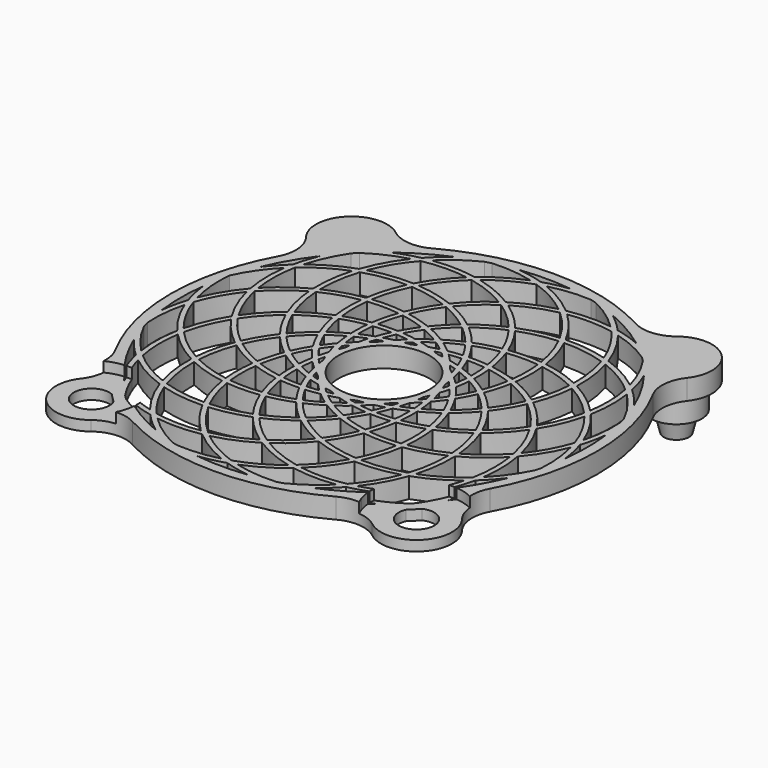
from build123d import *

# Parameters (mm, degrees)
F0_R          = 4.5
F0_R_2        = 2.5
F1_DEPTH      = 1
F1_DEPTH_BACK = 1
F1_FACE_R     = 4.5
F1_FACE_R_2   = 2.5
F2_DEPTH      = 1
F0_R_3        = 1.75
F3_DEPTH      = 3.5
F3_DEPTH_BACK = 1
F4_DEPTH      = 5.5
F4_DEPTH_BACK = 1
F5_SIZE2      = 0.49999
F5_SIZE       = 1.99999
F5_2_SIZE2    = 0.49999
F5_2_SIZE     = 1.99999
F6_T1_DEPTH   = 1
F6_T3_DEPTH   = 1
F6_T8_DEPTH   = 8.6156015126
F6_S10_R      = 4.5
F6_T11_DEPTH  = 6
F6_T16_DEPTH  = 1
F6_S17_R      = 4.5
F6_T18_DEPTH  = 4
F6_T22_DEPTH  = 1
F6_S23_R      = 4.5
F6_T24_DEPTH  = 4
F6_T28_DEPTH  = 8.6156015126
F6_S30_R      = 4.5
F6_T31_DEPTH  = 6
F6_T36_DEPTH  = 1
F6_S37_R      = 4.5
F6_T38_DEPTH  = 4
F6_T42_DEPTH  = 1
F6_S43_R      = 4.5
F6_T44_DEPTH  = 4
F6_T48_DEPTH  = 8.6156015126
F6_S50_R      = 4.5
F6_T51_DEPTH  = 6
F6_T56_DEPTH  = 1
F6_S57_R      = 4.5
F6_T58_DEPTH  = 4
F6_T62_DEPTH  = 1
F6_S63_R      = 4.5
F6_T64_DEPTH  = 4
F6_T68_DEPTH  = 8.6156015126
F6_S70_R      = 4.5
F6_T71_DEPTH  = 6
F6_T76_DEPTH  = 1
F6_S77_R      = 4.5
F6_T78_DEPTH  = 4
F6_T82_DEPTH  = 1
F6_S83_R      = 4.5
F6_T84_DEPTH  = 4


# Not quite as in the source:
# - a fillet or chamfer that OpenCascade refuses, or shapes differently, is made with other operations: its cross-section is extruded or revolved along the edge and cut away or added
# - a fillet or chamfer is up to 0.001 mm smaller than in the source, because OpenCascade refuses the exact size


with BuildPart() as f1:
    # F0 (on Top) → F1 (new body, two sides)
    with BuildSketch(Plane.XY) as f1_sk:
        with BuildLine():
            ThreePointArc((-12.5937572472, 16.8046802528), (-18.4748737342, 18.4748737342), (-16.8046802528, 12.5937572472))
            ThreePointArc((-16.8046802528, 12.5937572472), (-20.9933078109, 0.5301199445), (-17.4188888235, -11.7295486765))
            ThreePointArc((-17.4188888235, -11.7295486765), (-16.8926298485, -11.5894204515), (-16.3532972876, -11.5138902124))
            ThreePointArc((-16.3532972876, -11.5138902124), (-17.4969164616, -9.6880294351), (-18.4375, -7.7497479798))
            ThreePointArc((-18.4375, -7.7497479798), (-17.6217859595, -8.7419239844), (-16.7121426428, -9.6487600536))
            ThreePointArc((-16.7121426428, -9.6487600536), (-16.4747739333, -10.586073555), (-16.1683953277, -11.5031518801))
            ThreePointArc((-16.1683953277, -11.5031518801), (-15.8979515735, -11.5011572467), (-15.6278764222, -11.5154126117))
            ThreePointArc((-15.6278764222, -11.5154126117), (-15.8650198757, -10.8615610006), (-16.0654285483, -10.1955314885))
            ThreePointArc((-16.0654285483, -10.1955314885), (-14.2580516563, -11.3945947478), (-12.2764726786, -12.2764726786))
            ThreePointArc((-12.2764726786, -12.2764726786), (-11.3945947478, -14.2580516563), (-10.1955314885, -16.0654285483))
            ThreePointArc((-10.1955314885, -16.0654285483), (-10.8615610006, -15.8650198757), (-11.5154126117, -15.6278764222))
            ThreePointArc((-11.5154126117, -15.6278764222), (-11.503854804, -15.8137786896), (-11.5, -16))
            ThreePointArc((-11.5, -16), (-11.500788039, -16.0842124111), (-11.5031518801, -16.1683953277))
            ThreePointArc((-11.5031518801, -16.1683953277), (-10.586073555, -16.4747739333), (-9.6487600536, -16.7121426428))
            ThreePointArc((-9.6487600536, -16.7121426428), (-8.7419239844, -17.6217859595), (-7.7497479798, -18.4375))
            ThreePointArc((-7.7497479798, -18.4375), (-9.6880294351, -17.4969164616), (-11.5138902124, -16.3532972876))
            ThreePointArc((-11.5138902124, -16.3532972876), (-11.5894204515, -16.8926298485), (-11.7295486765, -17.4188888235))
            ThreePointArc((-11.7295486765, -17.4188888235), (0, -21), (11.7295486765, -17.4188888235))
            ThreePointArc((11.7295486765, -17.4188888235), (11.5894204515, -16.8926298485), (11.5138902124, -16.3532972876))
            ThreePointArc((11.5138902124, -16.3532972876), (9.6880294351, -17.4969164616), (7.7497479798, -18.4375))
            ThreePointArc((7.7497479798, -18.4375), (8.7419239844, -17.6217859595), (9.6487600536, -16.7121426428))
            ThreePointArc((9.6487600536, -16.7121426428), (10.586073555, -16.4747739333), (11.5031518801, -16.1683953277))
            ThreePointArc((11.5031518801, -16.1683953277), (11.5011572467, -15.8979515735), (11.5154126117, -15.6278764222))
            ThreePointArc((11.5154126117, -15.6278764222), (10.8615610006, -15.8650198757), (10.1955314885, -16.0654285483))
            ThreePointArc((10.1955314885, -16.0654285483), (11.3945947478, -14.2580516563), (12.2764726786, -12.2764726786))
            ThreePointArc((12.2764726786, -12.2764726786), (14.2580516563, -11.3945947478), (16.0654285483, -10.1955314885))
            ThreePointArc((16.0654285483, -10.1955314885), (15.8650198757, -10.8615610006), (15.6278764222, -11.5154126117))
            ThreePointArc((15.6278764222, -11.5154126117), (15.8979515735, -11.5011572467), (16.1683953277, -11.5031518801))
            ThreePointArc((16.1683953277, -11.5031518801), (16.4747739333, -10.586073555), (16.7121426428, -9.6487600536))
            ThreePointArc((16.7121426428, -9.6487600536), (17.6217859595, -8.7419239844), (18.4375, -7.7497479798))
            ThreePointArc((18.4375, -7.7497479798), (17.4969164616, -9.6880294351), (16.3532972876, -11.5138902124))
            ThreePointArc((16.3532972876, -11.5138902124), (16.8926298485, -11.5894204515), (17.4188888235, -11.7295486765))
            ThreePointArc((17.4188888235, -11.7295486765), (20.9933078109, 0.5301199445), (16.8046802528, 12.5937572472))
            ThreePointArc((16.8046802528, 12.5937572472), (18.4748737342, 18.4748737342), (12.5937572472, 16.8046802528))
            ThreePointArc((12.5937572472, 16.8046802528), (0, 21), (-12.5937572472, 16.8046802528))
        make_face()
        with BuildLine():
            ThreePointArc((-0.796875, -19.0108349897), (-2.8178445863, -19.3721780204), (-4.8707031411, -19.3978413982))
            ThreePointArc((-4.8707031411, -19.3978413982), (-5.1763809021, -19.3185165258), (-5.4807680447, -19.234375))
            ThreePointArc((-5.4807680447, -19.234375), (-7.2457640145, -18.1857205855), (-8.8153035012, -16.8623035483))
            ThreePointArc((-8.8153035012, -16.8623035483), (-6.6505375689, -16.9970343456), (-4.4935008692, -16.7699735479))
            ThreePointArc((-4.4935008692, -16.7699735479), (-2.7389826893, -18.0451323167), (-0.796875, -19.0108349897))
        make_face(mode=Mode.SUBTRACT)
        with BuildLine():
            ThreePointArc((-9.3854612563, -16.2560957484), (-10.6982047122, -14.4651694437), (-11.6733496354, -12.4702246354))
            ThreePointArc((-11.6733496354, -12.4702246354), (-9.6078487655, -12.9001869113), (-7.5, -12.9903810568))
            ThreePointArc((-7.5, -12.9903810568), (-6.367965196, -14.7707345623), (-4.9628565074, -16.3445296492))
            ThreePointArc((-4.9628565074, -16.3445296492), (-7.1781018522, -16.4975017775), (-9.3854612563, -16.2560957484))
        make_face(mode=Mode.SUBTRACT)
        with BuildLine():
            ThreePointArc((-8.3397829584, -8.9231359457), (-6.7301072697, -8.9984906043), (-5.123475383, -8.8741196746))
            ThreePointArc((-5.123475383, -8.8741196746), (-4.4278678242, -10.3276891679), (-3.5577709312, -11.6840318769))
            ThreePointArc((-3.5577709312, -11.6840318769), (-5.3503230612, -12.215940902), (-7.2021630117, -12.4745122606))
            ThreePointArc((-7.2021630117, -12.4745122606), (-7.9041536216, -10.7414861404), (-8.3397829584, -8.9231359457))
        make_face(mode=Mode.SUBTRACT)
        with BuildLine():
            ThreePointArc((-3.2416059412, -12.0978380705), (-1.9464668908, -13.4994857883), (-0.4600759958, -14.6964166934))
            ThreePointArc((-0.4600759958, -14.6964166934), (-2.3399691931, -15.6274721423), (-4.3490923933, -16.2310337785))
            ThreePointArc((-4.3490923933, -16.2310337785), (-5.7872633059, -14.7037724687), (-6.9497708467, -12.9575081989))
            ThreePointArc((-6.9497708467, -12.9575081989), (-5.0640531191, -12.6641310761), (-3.2416059412, -12.0978380705))
        make_face(mode=Mode.SUBTRACT)
        with BuildLine():
            ThreePointArc((-16.3445296492, -4.9628565074), (-14.7707345623, -6.367965196), (-12.9903810568, -7.5))
            ThreePointArc((-12.9903810568, -7.5), (-12.9001869113, -9.6078487655), (-12.4702246354, -11.6733496354))
            ThreePointArc((-12.4702246354, -11.6733496354), (-14.4651694437, -10.6982047122), (-16.2560957484, -9.3854612563))
            ThreePointArc((-16.2560957484, -9.3854612563), (-16.4975017775, -7.1781018522), (-16.3445296492, -4.9628565074))
        make_face(mode=Mode.SUBTRACT)
        with BuildLine():
            ThreePointArc((-12.4745122606, -7.2021630117), (-12.215940902, -5.3503230612), (-11.6840318769, -3.5577709312))
            ThreePointArc((-11.6840318769, -3.5577709312), (-10.3276891679, -4.4278678242), (-8.8741196746, -5.123475383))
            ThreePointArc((-8.8741196746, -5.123475383), (-8.9984906043, -6.7301072697), (-8.9231359457, -8.3397829584))
            ThreePointArc((-8.9231359457, -8.3397829584), (-10.7414861404, -7.9041536216), (-12.4745122606, -7.2021630117))
        make_face(mode=Mode.SUBTRACT)
        with BuildLine():
            ThreePointArc((-19.3978413982, -4.8707031411), (-19.3721780204, -2.8178445863), (-19.0108349897, -0.796875))
            ThreePointArc((-19.0108349897, -0.796875), (-18.0451323167, -2.7389826893), (-16.7699735479, -4.4935008692))
            ThreePointArc((-16.7699735479, -4.4935008692), (-16.9970343456, -6.6505375689), (-16.8623035483, -8.8153035012))
            ThreePointArc((-16.8623035483, -8.8153035012), (-18.1857205855, -7.2457640145), (-19.234375, -5.4807680447))
            ThreePointArc((-19.234375, -5.4807680447), (-19.3185165258, -5.1763809021), (-19.3978413982, -4.8707031411))
        make_face(mode=Mode.SUBTRACT)
        with BuildLine():
            ThreePointArc((-18.7709225126, 0), (-17.8763065644, 2.0323323338), (-16.6362061428, 3.8743050138))
            ThreePointArc((-16.6362061428, 3.8743050138), (-15.9758139615, 1.870547651), (-15, 0))
            ThreePointArc((-15, 0), (-15.9758139615, -1.870547651), (-16.6362061428, -3.8743050138))
            ThreePointArc((-16.6362061428, -3.8743050138), (-17.8763065644, -2.0323323338), (-18.7709225126, 0))
        make_face(mode=Mode.SUBTRACT)
        with BuildLine():
            ThreePointArc((-14.6964166934, -0.4600759958), (-13.4994857883, -1.9464668908), (-12.0978380705, -3.2416059412))
            ThreePointArc((-12.0978380705, -3.2416059412), (-12.6641310761, -5.0640531191), (-12.9575081989, -6.9497708467))
            ThreePointArc((-12.9575081989, -6.9497708467), (-14.7037724687, -5.7872633059), (-16.2310337785, -4.3490923933))
            ThreePointArc((-16.2310337785, -4.3490923933), (-15.6274721423, -2.3399691931), (-14.6964166934, -0.4600759958))
        make_face(mode=Mode.SUBTRACT)
        with BuildLine():
            ThreePointArc((-11.8975538896, -2.7608959312), (-13.2544766828, -1.4744547615), (-14.4043260233, 0))
            ThreePointArc((-14.4043260233, 0), (-13.2544766828, 1.4744547615), (-11.8975538896, 2.7608959312))
            ThreePointArc((-11.8975538896, 2.7608959312), (-11.1579750939, 1.3291985636), (-10.246950766, 0))
            ThreePointArc((-10.246950766, 0), (-11.1579750939, -1.3291985636), (-11.8975538896, -2.7608959312))
        make_face(mode=Mode.SUBTRACT)
        with BuildLine():
            ThreePointArc((-7.7466458467, -12.4974322032), (-9.8402088364, -12.3638032756), (-11.8819413852, -11.8819413852))
            ThreePointArc((-11.8819413852, -11.8819413852), (-12.3638032756, -9.8402088364), (-12.4974322032, -7.7466458467))
            ThreePointArc((-12.4974322032, -7.7466458467), (-10.7176641853, -8.4354326692), (-8.8562321294, -8.8562321294))
            ThreePointArc((-8.8562321294, -8.8562321294), (-8.4354326692, -10.7176641853), (-7.7466458467, -12.4974322032))
        make_face(mode=Mode.SUBTRACT)
        with BuildLine():
            ThreePointArc((-8.3943652328, -5.3065650226), (-7.1764321537, -5.6777588025), (-5.9280288991, -5.9280288991))
            ThreePointArc((-5.9280288991, -5.9280288991), (-5.6777588025, -7.1764321537), (-5.3065650226, -8.3943652328))
            ThreePointArc((-5.3065650226, -8.3943652328), (-6.8585742746, -8.4998060708), (-8.4116618732, -8.4116618732))
            ThreePointArc((-8.4116618732, -8.4116618732), (-8.4998060708, -6.8585742746), (-8.3943652328, -5.3065650226))
        make_face(mode=Mode.SUBTRACT)
        with BuildLine():
            ThreePointArc((-4.6164510289, -8.7928027328), (-3.3760931524, -8.5052994364), (-2.1698091714, -8.0978380705))
            ThreePointArc((-2.1698091714, -8.0978380705), (-1.3288672827, -9.0538519549), (-0.3984375, -9.9230160515))
            ThreePointArc((-0.3984375, -9.9230160515), (-1.6897965201, -10.7903351219), (-3.0788819336, -11.4905438068))
            ThreePointArc((-3.0788819336, -11.4905438068), (-3.9317608473, -10.1896025909), (-4.6164510289, -8.7928027328))
        make_face(mode=Mode.SUBTRACT)
        with BuildLine():
            ThreePointArc((-5.4115797281, -5.9949327154), (-4.4570283103, -6.0637606368), (-3.5, -6.0621778265))
            ThreePointArc((-3.5, -6.0621778265), (-3.0228565988, -6.8917800605), (-2.4859741615, -7.6840318769))
            ThreePointArc((-2.4859741615, -7.6840318769), (-3.6289007845, -8.0567244047), (-4.8023431781, -8.3179023798))
            ThreePointArc((-4.8023431781, -8.3179023798), (-5.1628776135, -7.1710824695), (-5.4115797281, -5.9949327154))
        make_face(mode=Mode.SUBTRACT)
        with BuildLine():
            ThreePointArc((-2.0070851639, -7.4905438068), (-2.5038687253, -6.7763369015), (-2.9497708467, -6.0293049687))
            ThreePointArc((-2.9497708467, -6.0293049687), (-2.2550131157, -5.9541498457), (-1.565297639, -5.8417703176))
            ThreePointArc((-1.565297639, -5.8417703176), (-1.0241762788, -6.2839515822), (-0.4600759958, -6.6964166934))
            ThreePointArc((-0.4600759958, -6.6964166934), (-1.2197545269, -7.1204142639), (-2.0070851639, -7.4905438068))
        make_face(mode=Mode.SUBTRACT)
        with BuildLine():
            ThreePointArc((-7.6840318769, -2.4859741615), (-6.8917800605, -3.0228565988), (-6.0621778265, -3.5))
            ThreePointArc((-6.0621778265, -3.5), (-6.0637606368, -4.4570283103), (-5.9949327154, -5.4115797281))
            ThreePointArc((-5.9949327154, -5.4115797281), (-7.1710824695, -5.1628776135), (-8.3179023798, -4.8023431781))
            ThreePointArc((-8.3179023798, -4.8023431781), (-8.0567244047, -3.6289007845), (-7.6840318769, -2.4859741615))
        make_face(mode=Mode.SUBTRACT)
        with BuildLine():
            ThreePointArc((-9.9230160515, -0.3984375), (-9.0538519549, -1.3288672827), (-8.0978380705, -2.1698091714))
            ThreePointArc((-8.0978380705, -2.1698091714), (-8.5052994364, -3.3760931524), (-8.7928027328, -4.6164510289))
            ThreePointArc((-8.7928027328, -4.6164510289), (-10.1896025909, -3.9317608473), (-11.4905438068, -3.0788819336))
            ThreePointArc((-11.4905438068, -3.0788819336), (-10.7903351219, -1.6897965201), (-9.9230160515, -0.3984375))
        make_face(mode=Mode.SUBTRACT)
        with BuildLine():
            ThreePointArc((-6.6964166934, -0.4600759958), (-6.2839515822, -1.0241762788), (-5.8417703176, -1.565297639))
            ThreePointArc((-5.8417703176, -1.565297639), (-5.9541498457, -2.2550131157), (-6.0293049687, -2.9497708467))
            ThreePointArc((-6.0293049687, -2.9497708467), (-6.7763369015, -2.5038687253), (-7.4905438068, -2.0070851639))
            ThreePointArc((-7.4905438068, -2.0070851639), (-7.1204142639, -1.2197545269), (-6.6964166934, -0.4600759958))
        make_face(mode=Mode.SUBTRACT)
        with BuildLine():
            ThreePointArc((-5.4834586429, -5.4834586429), (-5.5565823746, -4.6165455386), (-5.5692289729, -3.7466458467))
            ThreePointArc((-5.5692289729, -3.7466458467), (-4.9299735669, -4.0289384664), (-4.2764726786, -4.2764726786))
            ThreePointArc((-4.2764726786, -4.2764726786), (-4.0289384664, -4.9299735669), (-3.7466458467, -5.5692289729))
            ThreePointArc((-3.7466458467, -5.5692289729), (-4.6165455386, -5.5565823746), (-5.4834586429, -5.4834586429))
        make_face(mode=Mode.SUBTRACT)
        with BuildLine():
            ThreePointArc((-3.2021630117, -5.5463090303), (-3.4504043214, -5.0138050299), (-3.6733496354, -4.4702246354))
            ThreePointArc((-3.6733496354, -4.4702246354), (-3.199240696, -4.6001928148), (-2.7205568233, -4.7121426428))
            ThreePointArc((-2.7205568233, -4.7121426428), (-2.3842634919, -5.070720123), (-2.0346532772, -5.4163264189))
            ThreePointArc((-2.0346532772, -5.4163264189), (-2.6168803648, -5.4950403106), (-3.2021630117, -5.5463090303))
        make_face(mode=Mode.SUBTRACT)
        with BuildLine():
            ThreePointArc((-5.4163264189, -2.0346532772), (-5.070720123, -2.3842634919), (-4.7121426428, -2.7205568233))
            ThreePointArc((-4.7121426428, -2.7205568233), (-4.6001928148, -3.199240696), (-4.4702246354, -3.6733496354))
            ThreePointArc((-4.4702246354, -3.6733496354), (-5.0138050299, -3.4504043214), (-5.5463090303, -3.2021630117))
            ThreePointArc((-5.5463090303, -3.2021630117), (-5.4950403106, -2.6168803648), (-5.4163264189, -2.0346532772))
        make_face(mode=Mode.SUBTRACT)
        with BuildLine():
            ThreePointArc((-3.8819413852, -3.8819413852), (-3.9776278539, -3.5758119348), (-4.0654285483, -3.2673282582))
            ThreePointArc((-4.0654285483, -3.2673282582), (-3.8400676981, -3.4416250465), (-3.6109414404, -3.6109414404))
            ThreePointArc((-3.6109414404, -3.6109414404), (-3.4416250465, -3.8400676981), (-3.2673282582, -4.0654285483))
            ThreePointArc((-3.2673282582, -4.0654285483), (-3.5758119348, -3.9776278539), (-3.8819413852, -3.8819413852))
        make_face(mode=Mode.SUBTRACT)
        with BuildLine():
            ThreePointArc((-1.420889163, -5.3028305482), (-1.6568208009, -5.0855579017), (-1.8871002709, -4.8623035483))
            ThreePointArc((-1.8871002709, -4.8623035483), (-1.6047836555, -4.9005685696), (-1.3216962988, -4.9326377392))
            ThreePointArc((-1.3216962988, -4.9326377392), (-1.0605008715, -5.046408702), (-0.796875, -5.1544285292))
            ThreePointArc((-0.796875, -5.1544285292), (-1.1079300478, -5.2326327357), (-1.420889163, -5.3028305482))
        make_face(mode=Mode.SUBTRACT)
        with BuildLine():
            ThreePointArc((-4.8623035483, -1.8871002709), (-5.0855579017, -1.6568208009), (-5.3028305482, -1.420889163))
            ThreePointArc((-5.3028305482, -1.420889163), (-5.2326327357, -1.1079300478), (-5.1544285292, -0.796875))
            ThreePointArc((-5.1544285292, -0.796875), (-5.046408702, -1.0605008715), (-4.9326377392, -1.3216962988))
            ThreePointArc((-4.9326377392, -1.3216962988), (-4.9005685696, -1.6047836555), (-4.8623035483, -1.8871002709))
        make_face(mode=Mode.SUBTRACT)
        with BuildLine():
            ThreePointArc((2.5072713766, -19.8422173722), (0, -20), (-2.5072713766, -19.8422173722))
            ThreePointArc((-2.5072713766, -19.8422173722), (-1.2401647313, -19.6318762932), (0, -19.2975201071))
            ThreePointArc((0, -19.2975201071), (1.2401647313, -19.6318762932), (2.5072713766, -19.8422173722))
        make_face(mode=Mode.SUBTRACT)
        with BuildLine():
            ThreePointArc((0, -18.7709225126), (-2.0323323338, -17.8763065644), (-3.8743050138, -16.6362061428))
            ThreePointArc((-3.8743050138, -16.6362061428), (-1.870547651, -15.9758139615), (0, -15))
            ThreePointArc((0, -15), (1.870547651, -15.9758139615), (3.8743050138, -16.6362061428))
            ThreePointArc((3.8743050138, -16.6362061428), (2.0323323338, -17.8763065644), (0, -18.7709225126))
        make_face(mode=Mode.SUBTRACT)
        with BuildLine():
            ThreePointArc((8.8153035012, -16.8623035483), (7.2457640145, -18.1857205855), (5.4807680447, -19.234375))
            ThreePointArc((5.4807680447, -19.234375), (5.1763809021, -19.3185165258), (4.8707031411, -19.3978413982))
            ThreePointArc((4.8707031411, -19.3978413982), (2.8178445863, -19.3721780204), (0.796875, -19.0108349897))
            ThreePointArc((0.796875, -19.0108349897), (2.7389826893, -18.0451323167), (4.4935008692, -16.7699735479))
            ThreePointArc((4.4935008692, -16.7699735479), (6.6505375689, -16.9970343456), (8.8153035012, -16.8623035483))
        make_face(mode=Mode.SUBTRACT)
        with BuildLine():
            ThreePointArc((4.3490923933, -16.2310337785), (2.3399691931, -15.6274721423), (0.4600759958, -14.6964166934))
            ThreePointArc((0.4600759958, -14.6964166934), (1.9464668908, -13.4994857883), (3.2416059412, -12.0978380705))
            ThreePointArc((3.2416059412, -12.0978380705), (5.0640531191, -12.6641310761), (6.9497708467, -12.9575081989))
            ThreePointArc((6.9497708467, -12.9575081989), (5.7872633059, -14.7037724687), (4.3490923933, -16.2310337785))
        make_face(mode=Mode.SUBTRACT)
        with BuildLine():
            ThreePointArc((0, -14.4043260233), (-1.4744547615, -13.2544766828), (-2.7608959312, -11.8975538896))
            ThreePointArc((-2.7608959312, -11.8975538896), (-1.3291985636, -11.1579750939), (0, -10.246950766))
            ThreePointArc((0, -10.246950766), (1.3291985636, -11.1579750939), (2.7608959312, -11.8975538896))
            ThreePointArc((2.7608959312, -11.8975538896), (1.4744547615, -13.2544766828), (0, -14.4043260233))
        make_face(mode=Mode.SUBTRACT)
        with BuildLine():
            ThreePointArc((4.9628565074, -16.3445296492), (6.367965196, -14.7707345623), (7.5, -12.9903810568))
            ThreePointArc((7.5, -12.9903810568), (9.6078487655, -12.9001869113), (11.6733496354, -12.4702246354))
            ThreePointArc((11.6733496354, -12.4702246354), (10.6982047122, -14.4651694437), (9.3854612563, -16.2560957484))
            ThreePointArc((9.3854612563, -16.2560957484), (7.1781018522, -16.4975017775), (4.9628565074, -16.3445296492))
        make_face(mode=Mode.SUBTRACT)
        with BuildLine():
            ThreePointArc((7.2021630117, -12.4745122606), (5.3503230612, -12.215940902), (3.5577709312, -11.6840318769))
            ThreePointArc((3.5577709312, -11.6840318769), (4.4278678242, -10.3276891679), (5.123475383, -8.8741196746))
            ThreePointArc((5.123475383, -8.8741196746), (6.7301072697, -8.9984906043), (8.3397829584, -8.9231359457))
            ThreePointArc((8.3397829584, -8.9231359457), (7.9041536216, -10.7414861404), (7.2021630117, -12.4745122606))
        make_face(mode=Mode.SUBTRACT)
        with BuildLine():
            ThreePointArc((3.0788819336, -11.4905438068), (1.6897965201, -10.7903351219), (0.3984375, -9.9230160515))
            ThreePointArc((0.3984375, -9.9230160515), (1.3288672827, -9.0538519549), (2.1698091714, -8.0978380705))
            ThreePointArc((2.1698091714, -8.0978380705), (3.3760931524, -8.5052994364), (4.6164510289, -8.7928027328))
            ThreePointArc((4.6164510289, -8.7928027328), (3.9317608473, -10.1896025909), (3.0788819336, -11.4905438068))
        make_face(mode=Mode.SUBTRACT)
        with BuildLine():
            ThreePointArc((-1.6890991615, -7.8975538896), (-0.8280194237, -7.4798849091), (0, -7))
            ThreePointArc((0, -7), (0.8280194237, -7.4798849091), (1.6890991615, -7.8975538896))
            ThreePointArc((1.6890991615, -7.8975538896), (0.8856419352, -8.791778398), (0, -9.6046863561))
            ThreePointArc((0, -9.6046863561), (-0.8856419352, -8.791778398), (-1.6890991615, -7.8975538896))
        make_face(mode=Mode.SUBTRACT)
        with BuildLine():
            ThreePointArc((2.0070851639, -7.4905438068), (1.2197545269, -7.1204142639), (0.4600759958, -6.6964166934))
            ThreePointArc((0.4600759958, -6.6964166934), (1.0241762788, -6.2839515822), (1.565297639, -5.8417703176))
            ThreePointArc((1.565297639, -5.8417703176), (2.2550131157, -5.9541498457), (2.9497708467, -6.0293049687))
            ThreePointArc((2.9497708467, -6.0293049687), (2.5038687253, -6.7763369015), (2.0070851639, -7.4905438068))
        make_face(mode=Mode.SUBTRACT)
        with BuildLine():
            ThreePointArc((0, -6.4043260233), (-0.4812352807, -6.0672846862), (-0.9461017835, -5.7080029125))
            ThreePointArc((-0.9461017835, -5.7080029125), (-0.4705273082, -5.5835041879), (0, -5.4411136466))
            ThreePointArc((0, -5.4411136466), (0.4705273082, -5.5835041879), (0.9461017835, -5.7080029125))
            ThreePointArc((0.9461017835, -5.7080029125), (0.4812352807, -6.0672846862), (0, -6.4043260233))
        make_face(mode=Mode.SUBTRACT)
        with BuildLine():
            ThreePointArc((2.4859741615, -7.6840318769), (3.0228565988, -6.8917800605), (3.5, -6.0621778265))
            ThreePointArc((3.5, -6.0621778265), (4.4570283103, -6.0637606368), (5.4115797281, -5.9949327154))
            ThreePointArc((5.4115797281, -5.9949327154), (5.1628776135, -7.1710824695), (4.8023431781, -8.3179023798))
            ThreePointArc((4.8023431781, -8.3179023798), (3.6289007845, -8.0567244047), (2.4859741615, -7.6840318769))
        make_face(mode=Mode.SUBTRACT)
        with BuildLine():
            ThreePointArc((7.7466458467, -12.4974322032), (8.4354326692, -10.7176641853), (8.8562321294, -8.8562321294))
            ThreePointArc((8.8562321294, -8.8562321294), (10.7176641853, -8.4354326692), (12.4974322032, -7.7466458467))
            ThreePointArc((12.4974322032, -7.7466458467), (12.3638032756, -9.8402088364), (11.8819413852, -11.8819413852))
            ThreePointArc((11.8819413852, -11.8819413852), (9.8402088364, -12.3638032756), (7.7466458467, -12.4974322032))
        make_face(mode=Mode.SUBTRACT)
        with BuildLine():
            ThreePointArc((8.4116618732, -8.4116618732), (6.8585742746, -8.4998060708), (5.3065650226, -8.3943652328))
            ThreePointArc((5.3065650226, -8.3943652328), (5.6777588025, -7.1764321537), (5.9280288991, -5.9280288991))
            ThreePointArc((5.9280288991, -5.9280288991), (7.1764321537, -5.6777588025), (8.3943652328, -5.3065650226))
            ThreePointArc((8.3943652328, -5.3065650226), (8.4998060708, -6.8585742746), (8.4116618732, -8.4116618732))
        make_face(mode=Mode.SUBTRACT)
        with BuildLine():
            ThreePointArc((1.420889163, -5.3028305482), (1.1079300478, -5.2326327357), (0.796875, -5.1544285292))
            ThreePointArc((0.796875, -5.1544285292), (1.0605008715, -5.046408702), (1.3216962988, -4.9326377392))
            ThreePointArc((1.3216962988, -4.9326377392), (1.6047836555, -4.9005685696), (1.8871002709, -4.8623035483))
            ThreePointArc((1.8871002709, -4.8623035483), (1.6568208009, -5.0855579017), (1.420889163, -5.3028305482))
        make_face(mode=Mode.SUBTRACT)
        with BuildLine():
            ThreePointArc((3.2021630117, -5.5463090303), (2.6168803648, -5.4950403106), (2.0346532772, -5.4163264189))
            ThreePointArc((2.0346532772, -5.4163264189), (2.3842634919, -5.070720123), (2.7205568233, -4.7121426428))
            ThreePointArc((2.7205568233, -4.7121426428), (3.199240696, -4.6001928148), (3.6733496354, -4.4702246354))
            ThreePointArc((3.6733496354, -4.4702246354), (3.4504043214, -5.0138050299), (3.2021630117, -5.5463090303))
        make_face(mode=Mode.SUBTRACT)
        with BuildLine():
            ThreePointArc((3.7466458467, -5.5692289729), (4.0289384664, -4.9299735669), (4.2764726786, -4.2764726786))
            ThreePointArc((4.2764726786, -4.2764726786), (4.9299735669, -4.0289384664), (5.5692289729, -3.7466458467))
            ThreePointArc((5.5692289729, -3.7466458467), (5.5565823746, -4.6165455386), (5.4834586429, -5.4834586429))
            ThreePointArc((5.4834586429, -5.4834586429), (4.6165455386, -5.5565823746), (3.7466458467, -5.5692289729))
        make_face(mode=Mode.SUBTRACT)
        with BuildLine():
            ThreePointArc((3.8819413852, -3.8819413852), (3.5758119348, -3.9776278539), (3.2673282582, -4.0654285483))
            ThreePointArc((3.2673282582, -4.0654285483), (3.4416250465, -3.8400676981), (3.6109414404, -3.6109414404))
            ThreePointArc((3.6109414404, -3.6109414404), (3.8400676981, -3.4416250465), (4.0654285483, -3.2673282582))
            ThreePointArc((4.0654285483, -3.2673282582), (3.9776278539, -3.5758119348), (3.8819413852, -3.8819413852))
        make_face(mode=Mode.SUBTRACT)
        with BuildLine():
            ThreePointArc((5.5463090303, -3.2021630117), (5.0138050299, -3.4504043214), (4.4702246354, -3.6733496354))
            ThreePointArc((4.4702246354, -3.6733496354), (4.6001928148, -3.199240696), (4.7121426428, -2.7205568233))
            ThreePointArc((4.7121426428, -2.7205568233), (5.070720123, -2.3842634919), (5.4163264189, -2.0346532772))
            ThreePointArc((5.4163264189, -2.0346532772), (5.4950403106, -2.6168803648), (5.5463090303, -3.2021630117))
        make_face(mode=Mode.SUBTRACT)
        Circle(F0_R, mode=Mode.SUBTRACT)
        with BuildLine():
            ThreePointArc((5.3028305482, -1.420889163), (5.0855579017, -1.6568208009), (4.8623035483, -1.8871002709))
            ThreePointArc((4.8623035483, -1.8871002709), (4.9005685696, -1.6047836555), (4.9326377392, -1.3216962988))
            ThreePointArc((4.9326377392, -1.3216962988), (5.046408702, -1.0605008715), (5.1544285292, -0.796875))
            ThreePointArc((5.1544285292, -0.796875), (5.2326327357, -1.1079300478), (5.3028305482, -1.420889163))
        make_face(mode=Mode.SUBTRACT)
        with BuildLine():
            ThreePointArc((7.6840318769, -2.4859741615), (8.0567244047, -3.6289007845), (8.3179023798, -4.8023431781))
            ThreePointArc((8.3179023798, -4.8023431781), (7.1710824695, -5.1628776135), (5.9949327154, -5.4115797281))
            ThreePointArc((5.9949327154, -5.4115797281), (6.0637606368, -4.4570283103), (6.0621778265, -3.5))
            ThreePointArc((6.0621778265, -3.5), (6.8917800605, -3.0228565988), (7.6840318769, -2.4859741615))
        make_face(mode=Mode.SUBTRACT)
        with BuildLine():
            ThreePointArc((6.6964166934, -0.4600759958), (7.1204142639, -1.2197545269), (7.4905438068, -2.0070851639))
            ThreePointArc((7.4905438068, -2.0070851639), (6.7763369015, -2.5038687253), (6.0293049687, -2.9497708467))
            ThreePointArc((6.0293049687, -2.9497708467), (5.9541498457, -2.2550131157), (5.8417703176, -1.565297639))
            ThreePointArc((5.8417703176, -1.565297639), (6.2839515822, -1.0241762788), (6.6964166934, -0.4600759958))
        make_face(mode=Mode.SUBTRACT)
        with BuildLine():
            ThreePointArc((5.7080029125, -0.9461017835), (5.5835041879, -0.4705273082), (5.4411136466, 0))
            ThreePointArc((5.4411136466, 0), (5.5835041879, 0.4705273082), (5.7080029125, 0.9461017835))
            ThreePointArc((5.7080029125, 0.9461017835), (6.0672846862, 0.4812352807), (6.4043260233, 0))
            ThreePointArc((6.4043260233, 0), (6.0672846862, -0.4812352807), (5.7080029125, -0.9461017835))
        make_face(mode=Mode.SUBTRACT)
        with BuildLine():
            ThreePointArc((11.4905438068, -3.0788819336), (10.1896025909, -3.9317608473), (8.7928027328, -4.6164510289))
            ThreePointArc((8.7928027328, -4.6164510289), (8.5052994364, -3.3760931524), (8.0978380705, -2.1698091714))
            ThreePointArc((8.0978380705, -2.1698091714), (9.0538519549, -1.3288672827), (9.9230160515, -0.3984375))
            ThreePointArc((9.9230160515, -0.3984375), (10.7903351219, -1.6897965201), (11.4905438068, -3.0788819336))
        make_face(mode=Mode.SUBTRACT)
        with BuildLine():
            ThreePointArc((7.8975538896, -1.6890991615), (7.4798849091, -0.8280194237), (7, 0))
            ThreePointArc((7, 0), (7.4798849091, 0.8280194237), (7.8975538896, 1.6890991615))
            ThreePointArc((7.8975538896, 1.6890991615), (8.791778398, 0.8856419352), (9.6046863561, 0))
            ThreePointArc((9.6046863561, 0), (8.791778398, -0.8856419352), (7.8975538896, -1.6890991615))
        make_face(mode=Mode.SUBTRACT)
        with BuildLine():
            ThreePointArc((12.4702246354, -11.6733496354), (12.9001869113, -9.6078487655), (12.9903810568, -7.5))
            ThreePointArc((12.9903810568, -7.5), (14.7707345623, -6.367965196), (16.3445296492, -4.9628565074))
            ThreePointArc((16.3445296492, -4.9628565074), (16.4975017775, -7.1781018522), (16.2560957484, -9.3854612563))
            ThreePointArc((16.2560957484, -9.3854612563), (14.4651694437, -10.6982047122), (12.4702246354, -11.6733496354))
        make_face(mode=Mode.SUBTRACT)
        with BuildLine():
            ThreePointArc((11.6840318769, -3.5577709312), (12.215940902, -5.3503230612), (12.4745122606, -7.2021630117))
            ThreePointArc((12.4745122606, -7.2021630117), (10.7414861404, -7.9041536216), (8.9231359457, -8.3397829584))
            ThreePointArc((8.9231359457, -8.3397829584), (8.9984906043, -6.7301072697), (8.8741196746, -5.123475383))
            ThreePointArc((8.8741196746, -5.123475383), (10.3276891679, -4.4278678242), (11.6840318769, -3.5577709312))
        make_face(mode=Mode.SUBTRACT)
        with BuildLine():
            ThreePointArc((16.2310337785, -4.3490923933), (14.7037724687, -5.7872633059), (12.9575081989, -6.9497708467))
            ThreePointArc((12.9575081989, -6.9497708467), (12.6641310761, -5.0640531191), (12.0978380705, -3.2416059412))
            ThreePointArc((12.0978380705, -3.2416059412), (13.4994857883, -1.9464668908), (14.6964166934, -0.4600759958))
            ThreePointArc((14.6964166934, -0.4600759958), (15.6274721423, -2.3399691931), (16.2310337785, -4.3490923933))
        make_face(mode=Mode.SUBTRACT)
        with BuildLine():
            ThreePointArc((11.8975538896, -2.7608959312), (11.1579750939, -1.3291985636), (10.246950766, 0))
            ThreePointArc((10.246950766, 0), (11.1579750939, 1.3291985636), (11.8975538896, 2.7608959312))
            ThreePointArc((11.8975538896, 2.7608959312), (13.2544766828, 1.4744547615), (14.4043260233, 0))
            ThreePointArc((14.4043260233, 0), (13.2544766828, -1.4744547615), (11.8975538896, -2.7608959312))
        make_face(mode=Mode.SUBTRACT)
        with BuildLine():
            ThreePointArc((19.0108349897, -0.796875), (19.3721780204, -2.8178445863), (19.3978413982, -4.8707031411))
            ThreePointArc((19.3978413982, -4.8707031411), (19.3185165258, -5.1763809021), (19.234375, -5.4807680447))
            ThreePointArc((19.234375, -5.4807680447), (18.1857205855, -7.2457640145), (16.8623035483, -8.8153035012))
            ThreePointArc((16.8623035483, -8.8153035012), (16.9970343456, -6.6505375689), (16.7699735479, -4.4935008692))
            ThreePointArc((16.7699735479, -4.4935008692), (18.0451323167, -2.7389826893), (19.0108349897, -0.796875))
        make_face(mode=Mode.SUBTRACT)
        with BuildLine():
            ThreePointArc((18.7709225126, 0), (17.8763065644, -2.0323323338), (16.6362061428, -3.8743050138))
            ThreePointArc((16.6362061428, -3.8743050138), (15.9758139615, -1.870547651), (15, 0))
            ThreePointArc((15, 0), (15.9758139615, 1.870547651), (16.6362061428, 3.8743050138))
            ThreePointArc((16.6362061428, 3.8743050138), (17.8763065644, 2.0323323338), (18.7709225126, 0))
        make_face(mode=Mode.SUBTRACT)
        with BuildLine():
            ThreePointArc((19.8422173722, 2.5072713766), (20, 0), (19.8422173722, -2.5072713766))
            ThreePointArc((19.8422173722, -2.5072713766), (19.6318762932, -1.2401647313), (19.2975201071, 0))
            ThreePointArc((19.2975201071, 0), (19.6318762932, 1.2401647313), (19.8422173722, 2.5072713766))
        make_face(mode=Mode.SUBTRACT)
        with BuildLine():
            ThreePointArc((-19.8422173722, -2.5072713766), (-20, 0), (-19.8422173722, 2.5072713766))
            ThreePointArc((-19.8422173722, 2.5072713766), (-19.6318762932, 1.2401647313), (-19.2975201071, 0))
            ThreePointArc((-19.2975201071, 0), (-19.6318762932, -1.2401647313), (-19.8422173722, -2.5072713766))
        make_face(mode=Mode.SUBTRACT)
        with BuildLine():
            ThreePointArc((-19.0108349897, 0.796875), (-19.3863283993, 2.9776902262), (-19.3713781581, 5.1905451337))
            ThreePointArc((-19.3713781581, 5.1905451337), (-18.277897993, 7.1144088191), (-16.8623035483, 8.8153035012))
            ThreePointArc((-16.8623035483, 8.8153035012), (-16.9970343456, 6.6505375689), (-16.7699735479, 4.4935008692))
            ThreePointArc((-16.7699735479, 4.4935008692), (-18.0451323167, 2.7389826893), (-19.0108349897, 0.796875))
        make_face(mode=Mode.SUBTRACT)
        with BuildLine():
            ThreePointArc((-14.6964166934, 0.4600759958), (-15.6274721423, 2.3399691931), (-16.2310337785, 4.3490923933))
            ThreePointArc((-16.2310337785, 4.3490923933), (-14.7037724687, 5.7872633059), (-12.9575081989, 6.9497708467))
            ThreePointArc((-12.9575081989, 6.9497708467), (-12.6641310761, 5.0640531191), (-12.0978380705, 3.2416059412))
            ThreePointArc((-12.0978380705, 3.2416059412), (-13.4994857883, 1.9464668908), (-14.6964166934, 0.4600759958))
        make_face(mode=Mode.SUBTRACT)
        with BuildLine():
            ThreePointArc((-18.4375, 7.7497479798), (-17.3205080757, 10), (-15.9302286234, 12.0924693924))
            ThreePointArc((-15.9302286234, 12.0924693924), (-16.3816212282, 10.8899523088), (-16.7121426428, 9.6487600536))
            ThreePointArc((-16.7121426428, 9.6487600536), (-17.6217859595, 8.7419239844), (-18.4375, 7.7497479798))
        make_face(mode=Mode.SUBTRACT)
        with BuildLine():
            ThreePointArc((-11.6840318769, 3.5577709312), (-12.215940902, 5.3503230612), (-12.4745122606, 7.2021630117))
            ThreePointArc((-12.4745122606, 7.2021630117), (-10.7414861404, 7.9041536216), (-8.9231359457, 8.3397829584))
            ThreePointArc((-8.9231359457, 8.3397829584), (-8.9984906043, 6.7301072697), (-8.8741196746, 5.123475383))
            ThreePointArc((-8.8741196746, 5.123475383), (-10.3276891679, 4.4278678242), (-11.6840318769, 3.5577709312))
        make_face(mode=Mode.SUBTRACT)
        with BuildLine():
            ThreePointArc((-12.9903810568, 7.5), (-14.7707345623, 6.367965196), (-16.3445296492, 4.9628565074))
            ThreePointArc((-16.3445296492, 4.9628565074), (-16.4975017775, 7.1781018522), (-16.2560957484, 9.3854612563))
            ThreePointArc((-16.2560957484, 9.3854612563), (-14.4651694437, 10.6982047122), (-12.4702246354, 11.6733496354))
            ThreePointArc((-12.4702246354, 11.6733496354), (-12.9001869113, 9.6078487655), (-12.9903810568, 7.5))
        make_face(mode=Mode.SUBTRACT)
        with BuildLine():
            ThreePointArc((-7.8975538896, 1.6890991615), (-7.4798849091, 0.8280194237), (-7, 0))
            ThreePointArc((-7, 0), (-7.4798849091, -0.8280194237), (-7.8975538896, -1.6890991615))
            ThreePointArc((-7.8975538896, -1.6890991615), (-8.791778398, -0.8856419352), (-9.6046863561, 0))
            ThreePointArc((-9.6046863561, 0), (-8.791778398, 0.8856419352), (-7.8975538896, 1.6890991615))
        make_face(mode=Mode.SUBTRACT)
        with BuildLine():
            ThreePointArc((-11.4905438068, 3.0788819336), (-10.1896025909, 3.9317608473), (-8.7928027328, 4.6164510289))
            ThreePointArc((-8.7928027328, 4.6164510289), (-8.5052994364, 3.3760931524), (-8.0978380705, 2.1698091714))
            ThreePointArc((-8.0978380705, 2.1698091714), (-9.0538519549, 1.3288672827), (-9.9230160515, 0.3984375))
            ThreePointArc((-9.9230160515, 0.3984375), (-10.7903351219, 1.6897965201), (-11.4905438068, 3.0788819336))
        make_face(mode=Mode.SUBTRACT)
        with BuildLine():
            ThreePointArc((-6.4043260233, 0), (-6.0672846862, 0.4812352807), (-5.7080029125, 0.9461017835))
            ThreePointArc((-5.7080029125, 0.9461017835), (-5.5835041879, 0.4705273082), (-5.4411136466, 0))
            ThreePointArc((-5.4411136466, 0), (-5.5835041879, -0.4705273082), (-5.7080029125, -0.9461017835))
            ThreePointArc((-5.7080029125, -0.9461017835), (-6.0672846862, -0.4812352807), (-6.4043260233, 0))
        make_face(mode=Mode.SUBTRACT)
        with BuildLine():
            ThreePointArc((-6.0293049687, 2.9497708467), (-5.9541498457, 2.2550131157), (-5.8417703176, 1.565297639))
            ThreePointArc((-5.8417703176, 1.565297639), (-6.2839515822, 1.0241762788), (-6.6964166934, 0.4600759958))
            ThreePointArc((-6.6964166934, 0.4600759958), (-7.1204142639, 1.2197545269), (-7.4905438068, 2.0070851639))
            ThreePointArc((-7.4905438068, 2.0070851639), (-6.7763369015, 2.5038687253), (-6.0293049687, 2.9497708467))
        make_face(mode=Mode.SUBTRACT)
        with BuildLine():
            ThreePointArc((-5.9949327154, 5.4115797281), (-6.0637606368, 4.4570283103), (-6.0621778265, 3.5))
            ThreePointArc((-6.0621778265, 3.5), (-6.8917800605, 3.0228565988), (-7.6840318769, 2.4859741615))
            ThreePointArc((-7.6840318769, 2.4859741615), (-8.0567244047, 3.6289007845), (-8.3179023798, 4.8023431781))
            ThreePointArc((-8.3179023798, 4.8023431781), (-7.1710824695, 5.1628776135), (-5.9949327154, 5.4115797281))
        make_face(mode=Mode.SUBTRACT)
        with BuildLine():
            ThreePointArc((-5.1544285292, 0.796875), (-5.2326327357, 1.1079300478), (-5.3028305482, 1.420889163))
            ThreePointArc((-5.3028305482, 1.420889163), (-5.0855579017, 1.6568208009), (-4.8623035483, 1.8871002709))
            ThreePointArc((-4.8623035483, 1.8871002709), (-4.9005685696, 1.6047836555), (-4.9326377392, 1.3216962988))
            ThreePointArc((-4.9326377392, 1.3216962988), (-5.046408702, 1.0605008715), (-5.1544285292, 0.796875))
        make_face(mode=Mode.SUBTRACT)
        with BuildLine():
            ThreePointArc((-4.4702246354, 3.6733496354), (-4.6001928148, 3.199240696), (-4.7121426428, 2.7205568233))
            ThreePointArc((-4.7121426428, 2.7205568233), (-5.070720123, 2.3842634919), (-5.4163264189, 2.0346532772))
            ThreePointArc((-5.4163264189, 2.0346532772), (-5.4950403106, 2.6168803648), (-5.5463090303, 3.2021630117))
            ThreePointArc((-5.5463090303, 3.2021630117), (-5.0138050299, 3.4504043214), (-4.4702246354, 3.6733496354))
        make_face(mode=Mode.SUBTRACT)
        with BuildLine():
            ThreePointArc((-3.8819413852, 3.8819413852), (-3.5758119348, 3.9776278539), (-3.2673282582, 4.0654285483))
            ThreePointArc((-3.2673282582, 4.0654285483), (-3.4416250465, 3.8400676981), (-3.6109414404, 3.6109414404))
            ThreePointArc((-3.6109414404, 3.6109414404), (-3.8400676981, 3.4416250465), (-4.0654285483, 3.2673282582))
            ThreePointArc((-4.0654285483, 3.2673282582), (-3.9776278539, 3.5758119348), (-3.8819413852, 3.8819413852))
        make_face(mode=Mode.SUBTRACT)
        with BuildLine():
            ThreePointArc((-3.7466458467, 5.5692289729), (-4.0289384664, 4.9299735669), (-4.2764726786, 4.2764726786))
            ThreePointArc((-4.2764726786, 4.2764726786), (-4.9299735669, 4.0289384664), (-5.5692289729, 3.7466458467))
            ThreePointArc((-5.5692289729, 3.7466458467), (-5.5565823746, 4.6165455386), (-5.4834586429, 5.4834586429))
            ThreePointArc((-5.4834586429, 5.4834586429), (-4.6165455386, 5.5565823746), (-3.7466458467, 5.5692289729))
        make_face(mode=Mode.SUBTRACT)
        with BuildLine():
            ThreePointArc((-2.0346532772, 5.4163264189), (-2.3842634919, 5.070720123), (-2.7205568233, 4.7121426428))
            ThreePointArc((-2.7205568233, 4.7121426428), (-3.199240696, 4.6001928148), (-3.6733496354, 4.4702246354))
            ThreePointArc((-3.6733496354, 4.4702246354), (-3.4504043214, 5.0138050299), (-3.2021630117, 5.5463090303))
            ThreePointArc((-3.2021630117, 5.5463090303), (-2.6168803648, 5.4950403106), (-2.0346532772, 5.4163264189))
        make_face(mode=Mode.SUBTRACT)
        with BuildLine():
            ThreePointArc((-1.8871002709, 4.8623035483), (-1.6568208009, 5.0855579017), (-1.420889163, 5.3028305482))
            ThreePointArc((-1.420889163, 5.3028305482), (-1.1079300478, 5.2326327357), (-0.796875, 5.1544285292))
            ThreePointArc((-0.796875, 5.1544285292), (-1.0605008715, 5.046408702), (-1.3216962988, 4.9326377392))
            ThreePointArc((-1.3216962988, 4.9326377392), (-1.6047836555, 4.9005685696), (-1.8871002709, 4.8623035483))
        make_face(mode=Mode.SUBTRACT)
        with BuildLine():
            ThreePointArc((-8.4116618732, 8.4116618732), (-6.8585742746, 8.4998060708), (-5.3065650226, 8.3943652328))
            ThreePointArc((-5.3065650226, 8.3943652328), (-5.6777588025, 7.1764321537), (-5.9280288991, 5.9280288991))
            ThreePointArc((-5.9280288991, 5.9280288991), (-7.1764321537, 5.6777588025), (-8.3943652328, 5.3065650226))
            ThreePointArc((-8.3943652328, 5.3065650226), (-8.4998060708, 6.8585742746), (-8.4116618732, 8.4116618732))
        make_face(mode=Mode.SUBTRACT)
        with BuildLine():
            ThreePointArc((-12.4974322032, 7.7466458467), (-12.3638032756, 9.8402088364), (-11.8819413852, 11.8819413852))
            ThreePointArc((-11.8819413852, 11.8819413852), (-9.8402088364, 12.3638032756), (-7.7466458467, 12.4974322032))
            ThreePointArc((-7.7466458467, 12.4974322032), (-8.4354326692, 10.7176641853), (-8.8562321294, 8.8562321294))
            ThreePointArc((-8.8562321294, 8.8562321294), (-10.7176641853, 8.4354326692), (-12.4974322032, 7.7466458467))
        make_face(mode=Mode.SUBTRACT)
        with BuildLine():
            ThreePointArc((-4.8023431781, 8.3179023798), (-3.6289007845, 8.0567244047), (-2.4859741615, 7.6840318769))
            ThreePointArc((-2.4859741615, 7.6840318769), (-3.0228565988, 6.8917800605), (-3.5, 6.0621778265))
            ThreePointArc((-3.5, 6.0621778265), (-4.4570283103, 6.0637606368), (-5.4115797281, 5.9949327154))
            ThreePointArc((-5.4115797281, 5.9949327154), (-5.1628776135, 7.1710824695), (-4.8023431781, 8.3179023798))
        make_face(mode=Mode.SUBTRACT)
        with BuildLine():
            ThreePointArc((-2.9497708467, 6.0293049687), (-2.5038687253, 6.7763369015), (-2.0070851639, 7.4905438068))
            ThreePointArc((-2.0070851639, 7.4905438068), (-1.2197545269, 7.1204142639), (-0.4600759958, 6.6964166934))
            ThreePointArc((-0.4600759958, 6.6964166934), (-1.0241762788, 6.2839515822), (-1.565297639, 5.8417703176))
            ThreePointArc((-1.565297639, 5.8417703176), (-2.2550131157, 5.9541498457), (-2.9497708467, 6.0293049687))
        make_face(mode=Mode.SUBTRACT)
        with BuildLine():
            ThreePointArc((-4.6164510289, 8.7928027328), (-3.9317608473, 10.1896025909), (-3.0788819336, 11.4905438068))
            ThreePointArc((-3.0788819336, 11.4905438068), (-1.6897965201, 10.7903351219), (-0.3984375, 9.9230160515))
            ThreePointArc((-0.3984375, 9.9230160515), (-1.3288672827, 9.0538519549), (-2.1698091714, 8.0978380705))
            ThreePointArc((-2.1698091714, 8.0978380705), (-3.3760931524, 8.5052994364), (-4.6164510289, 8.7928027328))
        make_face(mode=Mode.SUBTRACT)
        with BuildLine():
            ThreePointArc((-16.0654285483, 10.1955314885), (-15.3678759992, 12.1264140059), (-14.3636718589, 13.9170733536))
            ThreePointArc((-14.3636718589, 13.9170733536), (-14.1421356237, 14.1421356237), (-13.9170733536, 14.3636718589))
            ThreePointArc((-13.9170733536, 14.3636718589), (-12.1264140059, 15.3678759992), (-10.1955314885, 16.0654285483))
            ThreePointArc((-10.1955314885, 16.0654285483), (-11.3945947478, 14.2580516563), (-12.2764726786, 12.2764726786))
            ThreePointArc((-12.2764726786, 12.2764726786), (-14.2580516563, 11.3945947478), (-16.0654285483, 10.1955314885))
        make_face(mode=Mode.SUBTRACT)
        with Locations((-16, 16)):
            Circle(F0_R_2, mode=Mode.SUBTRACT)
        with BuildLine():
            ThreePointArc((-8.3397829584, 8.9231359457), (-7.9041536216, 10.7414861404), (-7.2021630117, 12.4745122606))
            ThreePointArc((-7.2021630117, 12.4745122606), (-5.3503230612, 12.215940902), (-3.5577709312, 11.6840318769))
            ThreePointArc((-3.5577709312, 11.6840318769), (-4.4278678242, 10.3276891679), (-5.123475383, 8.8741196746))
            ThreePointArc((-5.123475383, 8.8741196746), (-6.7301072697, 8.9984906043), (-8.3397829584, 8.9231359457))
        make_face(mode=Mode.SUBTRACT)
        with BuildLine():
            ThreePointArc((-4.9628565074, 16.3445296492), (-6.367965196, 14.7707345623), (-7.5, 12.9903810568))
            ThreePointArc((-7.5, 12.9903810568), (-9.6078487655, 12.9001869113), (-11.6733496354, 12.4702246354))
            ThreePointArc((-11.6733496354, 12.4702246354), (-10.6982047122, 14.4651694437), (-9.3854612563, 16.2560957484))
            ThreePointArc((-9.3854612563, 16.2560957484), (-7.1781018522, 16.4975017775), (-4.9628565074, 16.3445296492))
        make_face(mode=Mode.SUBTRACT)
        with BuildLine():
            ThreePointArc((-0.4600759958, 14.6964166934), (-1.9464668908, 13.4994857883), (-3.2416059412, 12.0978380705))
            ThreePointArc((-3.2416059412, 12.0978380705), (-5.0640531191, 12.6641310761), (-6.9497708467, 12.9575081989))
            ThreePointArc((-6.9497708467, 12.9575081989), (-5.7872633059, 14.7037724687), (-4.3490923933, 16.2310337785))
            ThreePointArc((-4.3490923933, 16.2310337785), (-2.3399691931, 15.6274721423), (-0.4600759958, 14.6964166934))
        make_face(mode=Mode.SUBTRACT)
        with BuildLine():
            ThreePointArc((-12.0924693924, 15.9302286234), (-10, 17.3205080757), (-7.7497479798, 18.4375))
            ThreePointArc((-7.7497479798, 18.4375), (-8.7419239844, 17.6217859595), (-9.6487600536, 16.7121426428))
            ThreePointArc((-9.6487600536, 16.7121426428), (-10.8899523088, 16.3816212282), (-12.0924693924, 15.9302286234))
        make_face(mode=Mode.SUBTRACT)
        with BuildLine():
            ThreePointArc((-8.8153035012, 16.8623035483), (-7.2457640145, 18.1857205855), (-5.4807680447, 19.234375))
            ThreePointArc((-5.4807680447, 19.234375), (-5.1763809021, 19.3185165258), (-4.8707031411, 19.3978413982))
            ThreePointArc((-4.8707031411, 19.3978413982), (-2.8178445863, 19.3721780204), (-0.796875, 19.0108349897))
            ThreePointArc((-0.796875, 19.0108349897), (-2.7389826893, 18.0451323167), (-4.4935008692, 16.7699735479))
            ThreePointArc((-4.4935008692, 16.7699735479), (-6.6505375689, 16.9970343456), (-8.8153035012, 16.8623035483))
        make_face(mode=Mode.SUBTRACT)
        with BuildLine():
            ThreePointArc((4.8623035483, 1.8871002709), (5.0855579017, 1.6568208009), (5.3028305482, 1.420889163))
            ThreePointArc((5.3028305482, 1.420889163), (5.2326327357, 1.1079300478), (5.1544285292, 0.796875))
            ThreePointArc((5.1544285292, 0.796875), (5.046408702, 1.0605008715), (4.9326377392, 1.3216962988))
            ThreePointArc((4.9326377392, 1.3216962988), (4.9005685696, 1.6047836555), (4.8623035483, 1.8871002709))
        make_face(mode=Mode.SUBTRACT)
        with BuildLine():
            ThreePointArc((0.796875, 5.1544285292), (1.1079300478, 5.2326327357), (1.420889163, 5.3028305482))
            ThreePointArc((1.420889163, 5.3028305482), (1.6568208009, 5.0855579017), (1.8871002709, 4.8623035483))
            ThreePointArc((1.8871002709, 4.8623035483), (1.6047836555, 4.9005685696), (1.3216962988, 4.9326377392))
            ThreePointArc((1.3216962988, 4.9326377392), (1.0605008715, 5.046408702), (0.796875, 5.1544285292))
        make_face(mode=Mode.SUBTRACT)
        with BuildLine():
            ThreePointArc((3.8819413852, 3.8819413852), (3.9776278539, 3.5758119348), (4.0654285483, 3.2673282582))
            ThreePointArc((4.0654285483, 3.2673282582), (3.8400676981, 3.4416250465), (3.6109414404, 3.6109414404))
            ThreePointArc((3.6109414404, 3.6109414404), (3.4416250465, 3.8400676981), (3.2673282582, 4.0654285483))
            ThreePointArc((3.2673282582, 4.0654285483), (3.5758119348, 3.9776278539), (3.8819413852, 3.8819413852))
        make_face(mode=Mode.SUBTRACT)
        with BuildLine():
            ThreePointArc((5.5463090303, 3.2021630117), (5.4950403106, 2.6168803648), (5.4163264189, 2.0346532772))
            ThreePointArc((5.4163264189, 2.0346532772), (5.070720123, 2.3842634919), (4.7121426428, 2.7205568233))
            ThreePointArc((4.7121426428, 2.7205568233), (4.6001928148, 3.199240696), (4.4702246354, 3.6733496354))
            ThreePointArc((4.4702246354, 3.6733496354), (5.0138050299, 3.4504043214), (5.5463090303, 3.2021630117))
        make_face(mode=Mode.SUBTRACT)
        with BuildLine():
            ThreePointArc((3.2021630117, 5.5463090303), (3.4504043214, 5.0138050299), (3.6733496354, 4.4702246354))
            ThreePointArc((3.6733496354, 4.4702246354), (3.199240696, 4.6001928148), (2.7205568233, 4.7121426428))
            ThreePointArc((2.7205568233, 4.7121426428), (2.3842634919, 5.070720123), (2.0346532772, 5.4163264189))
            ThreePointArc((2.0346532772, 5.4163264189), (2.6168803648, 5.4950403106), (3.2021630117, 5.5463090303))
        make_face(mode=Mode.SUBTRACT)
        with BuildLine():
            ThreePointArc((5.4834586429, 5.4834586429), (5.5565823746, 4.6165455386), (5.5692289729, 3.7466458467))
            ThreePointArc((5.5692289729, 3.7466458467), (4.9299735669, 4.0289384664), (4.2764726786, 4.2764726786))
            ThreePointArc((4.2764726786, 4.2764726786), (4.0289384664, 4.9299735669), (3.7466458467, 5.5692289729))
            ThreePointArc((3.7466458467, 5.5692289729), (4.6165455386, 5.5565823746), (5.4834586429, 5.4834586429))
        make_face(mode=Mode.SUBTRACT)
        with BuildLine():
            ThreePointArc((6.6964166934, 0.4600759958), (6.2839515822, 1.0241762788), (5.8417703176, 1.565297639))
            ThreePointArc((5.8417703176, 1.565297639), (5.9541498457, 2.2550131157), (6.0293049687, 2.9497708467))
            ThreePointArc((6.0293049687, 2.9497708467), (6.7763369015, 2.5038687253), (7.4905438068, 2.0070851639))
            ThreePointArc((7.4905438068, 2.0070851639), (7.1204142639, 1.2197545269), (6.6964166934, 0.4600759958))
        make_face(mode=Mode.SUBTRACT)
        with BuildLine():
            ThreePointArc((11.4905438068, 3.0788819336), (10.7903351219, 1.6897965201), (9.9230160515, 0.3984375))
            ThreePointArc((9.9230160515, 0.3984375), (9.0538519549, 1.3288672827), (8.0978380705, 2.1698091714))
            ThreePointArc((8.0978380705, 2.1698091714), (8.5052994364, 3.3760931524), (8.7928027328, 4.6164510289))
            ThreePointArc((8.7928027328, 4.6164510289), (10.1896025909, 3.9317608473), (11.4905438068, 3.0788819336))
        make_face(mode=Mode.SUBTRACT)
        with BuildLine():
            ThreePointArc((8.3179023798, 4.8023431781), (8.0567244047, 3.6289007845), (7.6840318769, 2.4859741615))
            ThreePointArc((7.6840318769, 2.4859741615), (6.8917800605, 3.0228565988), (6.0621778265, 3.5))
            ThreePointArc((6.0621778265, 3.5), (6.0637606368, 4.4570283103), (5.9949327154, 5.4115797281))
            ThreePointArc((5.9949327154, 5.4115797281), (7.1710824695, 5.1628776135), (8.3179023798, 4.8023431781))
        make_face(mode=Mode.SUBTRACT)
        with BuildLine():
            ThreePointArc((0.9461017835, 5.7080029125), (0.4705273082, 5.5835041879), (0, 5.4411136466))
            ThreePointArc((0, 5.4411136466), (-0.4705273082, 5.5835041879), (-0.9461017835, 5.7080029125))
            ThreePointArc((-0.9461017835, 5.7080029125), (-0.4812352807, 6.0672846862), (0, 6.4043260233))
            ThreePointArc((0, 6.4043260233), (0.4812352807, 6.0672846862), (0.9461017835, 5.7080029125))
        make_face(mode=Mode.SUBTRACT)
        with BuildLine():
            ThreePointArc((2.9497708467, 6.0293049687), (2.2550131157, 5.9541498457), (1.565297639, 5.8417703176))
            ThreePointArc((1.565297639, 5.8417703176), (1.0241762788, 6.2839515822), (0.4600759958, 6.6964166934))
            ThreePointArc((0.4600759958, 6.6964166934), (1.2197545269, 7.1204142639), (2.0070851639, 7.4905438068))
            ThreePointArc((2.0070851639, 7.4905438068), (2.5038687253, 6.7763369015), (2.9497708467, 6.0293049687))
        make_face(mode=Mode.SUBTRACT)
        with BuildLine():
            ThreePointArc((5.4115797281, 5.9949327154), (4.4570283103, 6.0637606368), (3.5, 6.0621778265))
            ThreePointArc((3.5, 6.0621778265), (3.0228565988, 6.8917800605), (2.4859741615, 7.6840318769))
            ThreePointArc((2.4859741615, 7.6840318769), (3.6289007845, 8.0567244047), (4.8023431781, 8.3179023798))
            ThreePointArc((4.8023431781, 8.3179023798), (5.1628776135, 7.1710824695), (5.4115797281, 5.9949327154))
        make_face(mode=Mode.SUBTRACT)
        with BuildLine():
            ThreePointArc((-1.6890991615, 7.8975538896), (-0.8856419352, 8.791778398), (0, 9.6046863561))
            ThreePointArc((0, 9.6046863561), (0.8856419352, 8.791778398), (1.6890991615, 7.8975538896))
            ThreePointArc((1.6890991615, 7.8975538896), (0.8280194237, 7.4798849091), (0, 7))
            ThreePointArc((0, 7), (-0.8280194237, 7.4798849091), (-1.6890991615, 7.8975538896))
        make_face(mode=Mode.SUBTRACT)
        with BuildLine():
            ThreePointArc((0.3984375, 9.9230160515), (1.6897965201, 10.7903351219), (3.0788819336, 11.4905438068))
            ThreePointArc((3.0788819336, 11.4905438068), (3.9317608473, 10.1896025909), (4.6164510289, 8.7928027328))
            ThreePointArc((4.6164510289, 8.7928027328), (3.3760931524, 8.5052994364), (2.1698091714, 8.0978380705))
            ThreePointArc((2.1698091714, 8.0978380705), (1.3288672827, 9.0538519549), (0.3984375, 9.9230160515))
        make_face(mode=Mode.SUBTRACT)
        with BuildLine():
            ThreePointArc((8.4116618732, 8.4116618732), (8.4998060708, 6.8585742746), (8.3943652328, 5.3065650226))
            ThreePointArc((8.3943652328, 5.3065650226), (7.1764321537, 5.6777588025), (5.9280288991, 5.9280288991))
            ThreePointArc((5.9280288991, 5.9280288991), (5.6777588025, 7.1764321537), (5.3065650226, 8.3943652328))
            ThreePointArc((5.3065650226, 8.3943652328), (6.8585742746, 8.4998060708), (8.4116618732, 8.4116618732))
        make_face(mode=Mode.SUBTRACT)
        with BuildLine():
            ThreePointArc((11.8819413852, 11.8819413852), (12.3638032756, 9.8402088364), (12.4974322032, 7.7466458467))
            ThreePointArc((12.4974322032, 7.7466458467), (10.7176641853, 8.4354326692), (8.8562321294, 8.8562321294))
            ThreePointArc((8.8562321294, 8.8562321294), (8.4354326692, 10.7176641853), (7.7466458467, 12.4974322032))
            ThreePointArc((7.7466458467, 12.4974322032), (9.8402088364, 12.3638032756), (11.8819413852, 11.8819413852))
        make_face(mode=Mode.SUBTRACT)
        with BuildLine():
            ThreePointArc((14.6964166934, 0.4600759958), (13.4994857883, 1.9464668908), (12.0978380705, 3.2416059412))
            ThreePointArc((12.0978380705, 3.2416059412), (12.6641310761, 5.0640531191), (12.9575081989, 6.9497708467))
            ThreePointArc((12.9575081989, 6.9497708467), (14.7037724687, 5.7872633059), (16.2310337785, 4.3490923933))
            ThreePointArc((16.2310337785, 4.3490923933), (15.6274721423, 2.3399691931), (14.6964166934, 0.4600759958))
        make_face(mode=Mode.SUBTRACT)
        with BuildLine():
            ThreePointArc((16.8623035483, 8.8153035012), (18.1857205855, 7.2457640145), (19.234375, 5.4807680447))
            ThreePointArc((19.234375, 5.4807680447), (19.3185165258, 5.1763809021), (19.3978413982, 4.8707031411))
            ThreePointArc((19.3978413982, 4.8707031411), (19.3721780204, 2.8178445863), (19.0108349897, 0.796875))
            ThreePointArc((19.0108349897, 0.796875), (18.0451323167, 2.7389826893), (16.7699735479, 4.4935008692))
            ThreePointArc((16.7699735479, 4.4935008692), (16.9970343456, 6.6505375689), (16.8623035483, 8.8153035012))
        make_face(mode=Mode.SUBTRACT)
        with BuildLine():
            ThreePointArc((11.6840318769, 3.5577709312), (10.3276891679, 4.4278678242), (8.8741196746, 5.123475383))
            ThreePointArc((8.8741196746, 5.123475383), (8.9984906043, 6.7301072697), (8.9231359457, 8.3397829584))
            ThreePointArc((8.9231359457, 8.3397829584), (10.7414861404, 7.9041536216), (12.4745122606, 7.2021630117))
            ThreePointArc((12.4745122606, 7.2021630117), (12.215940902, 5.3503230612), (11.6840318769, 3.5577709312))
        make_face(mode=Mode.SUBTRACT)
        with BuildLine():
            ThreePointArc((16.3445296492, 4.9628565074), (14.7707345623, 6.367965196), (12.9903810568, 7.5))
            ThreePointArc((12.9903810568, 7.5), (12.9001869113, 9.6078487655), (12.4702246354, 11.6733496354))
            ThreePointArc((12.4702246354, 11.6733496354), (14.4651694437, 10.6982047122), (16.2560957484, 9.3854612563))
            ThreePointArc((16.2560957484, 9.3854612563), (16.4975017775, 7.1781018522), (16.3445296492, 4.9628565074))
        make_face(mode=Mode.SUBTRACT)
        with BuildLine():
            ThreePointArc((15.9302286234, 12.0924693924), (17.3205080757, 10), (18.4375, 7.7497479798))
            ThreePointArc((18.4375, 7.7497479798), (17.6217859595, 8.7419239844), (16.7121426428, 9.6487600536))
            ThreePointArc((16.7121426428, 9.6487600536), (16.3816212282, 10.8899523088), (15.9302286234, 12.0924693924))
        make_face(mode=Mode.SUBTRACT)
        with BuildLine():
            ThreePointArc((2.7608959312, 11.8975538896), (1.3291985636, 11.1579750939), (0, 10.246950766))
            ThreePointArc((0, 10.246950766), (-1.3291985636, 11.1579750939), (-2.7608959312, 11.8975538896))
            ThreePointArc((-2.7608959312, 11.8975538896), (-1.4744547615, 13.2544766828), (0, 14.4043260233))
            ThreePointArc((0, 14.4043260233), (1.4744547615, 13.2544766828), (2.7608959312, 11.8975538896))
        make_face(mode=Mode.SUBTRACT)
        with BuildLine():
            ThreePointArc((4.3490923933, 16.2310337785), (5.7872633059, 14.7037724687), (6.9497708467, 12.9575081989))
            ThreePointArc((6.9497708467, 12.9575081989), (5.0640531191, 12.6641310761), (3.2416059412, 12.0978380705))
            ThreePointArc((3.2416059412, 12.0978380705), (1.9464668908, 13.4994857883), (0.4600759958, 14.6964166934))
            ThreePointArc((0.4600759958, 14.6964166934), (2.3399691931, 15.6274721423), (4.3490923933, 16.2310337785))
        make_face(mode=Mode.SUBTRACT)
        with BuildLine():
            ThreePointArc((3.5577709312, 11.6840318769), (5.3503230612, 12.215940902), (7.2021630117, 12.4745122606))
            ThreePointArc((7.2021630117, 12.4745122606), (7.9041536216, 10.7414861404), (8.3397829584, 8.9231359457))
            ThreePointArc((8.3397829584, 8.9231359457), (6.7301072697, 8.9984906043), (5.123475383, 8.8741196746))
            ThreePointArc((5.123475383, 8.8741196746), (4.4278678242, 10.3276891679), (3.5577709312, 11.6840318769))
        make_face(mode=Mode.SUBTRACT)
        with BuildLine():
            ThreePointArc((11.6733496354, 12.4702246354), (9.6078487655, 12.9001869113), (7.5, 12.9903810568))
            ThreePointArc((7.5, 12.9903810568), (6.367965196, 14.7707345623), (4.9628565074, 16.3445296492))
            ThreePointArc((4.9628565074, 16.3445296492), (7.1781018522, 16.4975017775), (9.3854612563, 16.2560957484))
            ThreePointArc((9.3854612563, 16.2560957484), (10.6982047122, 14.4651694437), (11.6733496354, 12.4702246354))
        make_face(mode=Mode.SUBTRACT)
        with BuildLine():
            ThreePointArc((3.8743050138, 16.6362061428), (1.870547651, 15.9758139615), (0, 15))
            ThreePointArc((0, 15), (-1.870547651, 15.9758139615), (-3.8743050138, 16.6362061428))
            ThreePointArc((-3.8743050138, 16.6362061428), (-2.0323323338, 17.8763065644), (0, 18.7709225126))
            ThreePointArc((0, 18.7709225126), (2.0323323338, 17.8763065644), (3.8743050138, 16.6362061428))
        make_face(mode=Mode.SUBTRACT)
        with BuildLine():
            ThreePointArc((0.796875, 19.0108349897), (2.8178445863, 19.3721780204), (4.8707031411, 19.3978413982))
            ThreePointArc((4.8707031411, 19.3978413982), (5.1763809021, 19.3185165258), (5.4807680447, 19.234375))
            ThreePointArc((5.4807680447, 19.234375), (7.2457640145, 18.1857205855), (8.8153035012, 16.8623035483))
            ThreePointArc((8.8153035012, 16.8623035483), (6.6505375689, 16.9970343456), (4.4935008692, 16.7699735479))
            ThreePointArc((4.4935008692, 16.7699735479), (2.7389826893, 18.0451323167), (0.796875, 19.0108349897))
        make_face(mode=Mode.SUBTRACT)
        with BuildLine():
            ThreePointArc((-2.5072713766, 19.8422173722), (0, 20), (2.5072713766, 19.8422173722))
            ThreePointArc((2.5072713766, 19.8422173722), (1.2401647313, 19.6318762932), (0, 19.2975201071))
            ThreePointArc((0, 19.2975201071), (-1.2401647313, 19.6318762932), (-2.5072713766, 19.8422173722))
        make_face(mode=Mode.SUBTRACT)
        with BuildLine():
            ThreePointArc((7.7497479798, 18.4375), (10, 17.3205080757), (12.0924693924, 15.9302286234))
            ThreePointArc((12.0924693924, 15.9302286234), (10.8899523088, 16.3816212282), (9.6487600536, 16.7121426428))
            ThreePointArc((9.6487600536, 16.7121426428), (8.7419239844, 17.6217859595), (7.7497479798, 18.4375))
        make_face(mode=Mode.SUBTRACT)
        with BuildLine():
            ThreePointArc((13.9170733536, 14.3636718589), (14.1421356237, 14.1421356237), (14.3636718589, 13.9170733536))
            ThreePointArc((14.3636718589, 13.9170733536), (15.3678759992, 12.1264140059), (16.0654285483, 10.1955314885))
            ThreePointArc((16.0654285483, 10.1955314885), (14.2580516563, 11.3945947478), (12.2764726786, 12.2764726786))
            ThreePointArc((12.2764726786, 12.2764726786), (11.3945947478, 14.2580516563), (10.1955314885, 16.0654285483))
            ThreePointArc((10.1955314885, 16.0654285483), (12.1264140059, 15.3678759992), (13.9170733536, 14.3636718589))
        make_face(mode=Mode.SUBTRACT)
        with Locations((16, 16)):
            Circle(F0_R_2, mode=Mode.SUBTRACT)
    extrude(amount=F1_DEPTH)
    extrude(f1_sk.sketch, amount=-F1_DEPTH_BACK)

    # F1_face (on face) + F0 (on Top) → F2 (join)
    with BuildSketch(Plane(origin=(0.0006932606, 1.3187707471, 1), x_dir=(1, 0, 0), z_dir=(0, 0, 1))):
        with BuildLine():
            ThreePointArc((17.4181955629, -13.0483194236), (20.9926145503, -0.7886508026), (16.8039869922, 11.2749865001))
            ThreePointArc((16.8039869922, 11.2749865001), (18.4741804736, 17.156102987), (12.5930639866, 15.4859095057))
            ThreePointArc((12.5930639866, 15.4859095057), (-0.0006932606, 19.6812292529), (-12.5944505078, 15.4859095057))
            ThreePointArc((-12.5944505078, 15.4859095057), (-18.4755669948, 17.156102987), (-16.8053735134, 11.2749865001))
            ThreePointArc((-16.8053735134, 11.2749865001), (-20.9940010715, -0.7886508026), (-17.4195820841, -13.0483194236))
            ThreePointArc((-17.4195820841, -13.0483194236), (-16.8933231091, -12.9081911986), (-16.3539905482, -12.8326609595))
            ThreePointArc((-16.3539905482, -12.8326609595), (-17.4976097222, -11.0068001823), (-18.4381932606, -9.0685187269))
            ThreePointArc((-18.4381932606, -9.0685187269), (-17.6224792201, -10.0606947315), (-16.7128359034, -10.9675308007))
            ThreePointArc((-16.7128359034, -10.9675308007), (-16.4754671939, -11.9048443021), (-16.1690885883, -12.8219226272))
            ThreePointArc((-16.1690885883, -12.8219226272), (-15.8986448341, -12.8199279938), (-15.6285696828, -12.8341833589))
            ThreePointArc((-15.6285696828, -12.8341833589), (-15.8657131363, -12.1803317477), (-16.0661218089, -11.5143022356))
            ThreePointArc((-16.0661218089, -11.5143022356), (-14.2587449169, -12.7133654949), (-12.2771659392, -13.5952434257))
            ThreePointArc((-12.2771659392, -13.5952434257), (-11.3952880084, -15.5768224034), (-10.1962247491, -17.3841992954))
            ThreePointArc((-10.1962247491, -17.3841992954), (-10.8622542612, -17.1837906228), (-11.5161058723, -16.9466471693))
            ThreePointArc((-11.5161058723, -16.9466471693), (-11.5018505073, -17.2167223206), (-11.5038451407, -17.4871660748))
            ThreePointArc((-11.5038451407, -17.4871660748), (-10.5867668156, -17.7935446804), (-9.6494533142, -18.0309133899))
            ThreePointArc((-9.6494533142, -18.0309133899), (-8.742617245, -18.9405567066), (-7.7504412404, -19.7562707471))
            ThreePointArc((-7.7504412404, -19.7562707471), (-9.6887226957, -18.8156872087), (-11.514583473, -17.6720680347))
            ThreePointArc((-11.514583473, -17.6720680347), (-11.5901137121, -18.2114005956), (-11.7302419371, -18.7376595706))
            ThreePointArc((-11.7302419371, -18.7376595706), (-0.0006932606, -22.3187707471), (11.7288554159, -18.7376595706))
            ThreePointArc((11.7288554159, -18.7376595706), (11.5887271909, -18.2114005956), (11.5131969518, -17.6720680347))
            ThreePointArc((11.5131969518, -17.6720680347), (9.6873361745, -18.8156872087), (7.7490547192, -19.7562707471))
            ThreePointArc((7.7490547192, -19.7562707471), (8.7412307238, -18.9405567066), (9.648066793, -18.0309133899))
            ThreePointArc((9.648066793, -18.0309133899), (10.5853802944, -17.7935446804), (11.5024586195, -17.4871660748))
            ThreePointArc((11.5024586195, -17.4871660748), (11.5004639861, -17.2167223206), (11.5147193511, -16.9466471693))
            ThreePointArc((11.5147193511, -16.9466471693), (10.86086774, -17.1837906228), (10.1948382279, -17.3841992954))
            ThreePointArc((10.1948382279, -17.3841992954), (11.3939014872, -15.5768224034), (12.275779418, -13.5952434257))
            ThreePointArc((12.275779418, -13.5952434257), (14.2573583957, -12.7133654949), (16.0647352877, -11.5143022356))
            ThreePointArc((16.0647352877, -11.5143022356), (15.8643266151, -12.1803317477), (15.6271831616, -12.8341833589))
            ThreePointArc((15.6271831616, -12.8341833589), (15.8972583129, -12.8199279938), (16.1677020671, -12.8219226272))
            ThreePointArc((16.1677020671, -12.8219226272), (16.4740806727, -11.9048443021), (16.7114493822, -10.9675308007))
            ThreePointArc((16.7114493822, -10.9675308007), (17.6210926989, -10.0606947315), (18.4368067394, -9.0685187269))
            ThreePointArc((18.4368067394, -9.0685187269), (17.496223201, -11.0068001823), (16.352604027, -12.8326609595))
            ThreePointArc((16.352604027, -12.8326609595), (16.8919365879, -12.9081911986), (17.4181955629, -13.0483194236))
        make_face()
        with BuildLine():
            ThreePointArc((-4.4941941298, -18.088744295), (-2.7396759499, -19.3639030638), (-0.7975682606, -20.3296057368))
            ThreePointArc((-0.7975682606, -20.3296057368), (-2.8185378469, -20.6909487675), (-4.8713964017, -20.7166121454))
            ThreePointArc((-4.8713964017, -20.7166121454), (-5.1770741626, -20.6372872729), (-5.4814613053, -20.5531457471))
            ThreePointArc((-5.4814613053, -20.5531457471), (-7.2464572751, -19.5044913326), (-8.8159967618, -18.1810742954))
            ThreePointArc((-8.8159967618, -18.1810742954), (-6.6512308295, -18.3158050927), (-4.4941941298, -18.088744295))
        make_face(mode=Mode.SUBTRACT)
        with BuildLine():
            ThreePointArc((-7.5006932606, -14.3091518039), (-6.3686584566, -16.0895053094), (-4.963549768, -17.6633003963))
            ThreePointArc((-4.963549768, -17.6633003963), (-7.1787951128, -17.8162725246), (-9.3861545169, -17.5748664955))
            ThreePointArc((-9.3861545169, -17.5748664955), (-10.6988979728, -15.7839401909), (-11.674042896, -13.7889953825))
            ThreePointArc((-11.674042896, -13.7889953825), (-9.6085420261, -14.2189576584), (-7.5006932606, -14.3091518039))
        make_face(mode=Mode.SUBTRACT)
        with BuildLine():
            ThreePointArc((-7.2028562723, -13.7932830077), (-7.9048468822, -12.0602568875), (-8.340476219, -10.2419066928))
            ThreePointArc((-8.340476219, -10.2419066928), (-6.7308005303, -10.3172613514), (-5.1241686436, -10.1928904218))
            ThreePointArc((-5.1241686436, -10.1928904218), (-4.4285610848, -11.646459915), (-3.5584641918, -13.002802624))
            ThreePointArc((-3.5584641918, -13.002802624), (-5.3510163218, -13.5347116491), (-7.2028562723, -13.7932830077))
        make_face(mode=Mode.SUBTRACT)
        with BuildLine():
            ThreePointArc((-4.3497856539, -17.5498045256), (-5.7879565665, -16.0225432158), (-6.9504641073, -14.2762789461))
            ThreePointArc((-6.9504641073, -14.2762789461), (-5.0647463797, -13.9829018232), (-3.2422992018, -13.4166088176))
            ThreePointArc((-3.2422992018, -13.4166088176), (-1.9471601514, -14.8182565354), (-0.4607692564, -16.0151874405))
            ThreePointArc((-0.4607692564, -16.0151874405), (-2.3406624537, -16.9462428894), (-4.3497856539, -17.5498045256))
        make_face(mode=Mode.SUBTRACT)
        with BuildLine():
            ThreePointArc((-16.256789009, -10.7042320034), (-16.4981950381, -8.4968725993), (-16.3452229098, -6.2816272546))
            ThreePointArc((-16.3452229098, -6.2816272546), (-14.7714278229, -7.6867359431), (-12.9910743174, -8.8187707471))
            ThreePointArc((-12.9910743174, -8.8187707471), (-12.9008801719, -10.9266195126), (-12.470917896, -12.9921203825))
            ThreePointArc((-12.470917896, -12.9921203825), (-14.4658627043, -12.0169754593), (-16.256789009, -10.7042320034))
        make_face(mode=Mode.SUBTRACT)
        with BuildLine():
            ThreePointArc((-8.9238292063, -9.6585537055), (-10.742179401, -9.2229243687), (-12.4752055212, -8.5209337588))
            ThreePointArc((-12.4752055212, -8.5209337588), (-12.2166341625, -6.6690938083), (-11.6847251375, -4.8765416783))
            ThreePointArc((-11.6847251375, -4.8765416783), (-10.3283824285, -5.7466385713), (-8.8748129352, -6.4422461301))
            ThreePointArc((-8.8748129352, -6.4422461301), (-8.9991838649, -8.0488780168), (-8.9238292063, -9.6585537055))
        make_face(mode=Mode.SUBTRACT)
        with BuildLine():
            ThreePointArc((-19.3985346588, -6.1894738882), (-19.372871281, -4.1366153335), (-19.0115282503, -2.1156457471))
            ThreePointArc((-19.0115282503, -2.1156457471), (-18.0458255773, -4.0577534364), (-16.7706668085, -5.8122716164))
            ThreePointArc((-16.7706668085, -5.8122716164), (-16.9977276062, -7.969308316), (-16.8629968089, -10.1340742483))
            ThreePointArc((-16.8629968089, -10.1340742483), (-18.1864138461, -8.5645347616), (-19.2350682606, -6.7995387918))
            ThreePointArc((-19.2350682606, -6.7995387918), (-19.3192097864, -6.4951516492), (-19.3985346588, -6.1894738882))
        make_face(mode=Mode.SUBTRACT)
        with BuildLine():
            ThreePointArc((-16.6368994034, -5.1930757609), (-17.876999825, -3.3511030809), (-18.7716157732, -1.3187707471))
            ThreePointArc((-18.7716157732, -1.3187707471), (-17.876999825, 0.7135615867), (-16.6368994034, 2.5555342667))
            ThreePointArc((-16.6368994034, 2.5555342667), (-15.9765072221, 0.5517769039), (-15.0006932606, -1.3187707471))
            ThreePointArc((-15.0006932606, -1.3187707471), (-15.9765072221, -3.1893183981), (-16.6368994034, -5.1930757609))
        make_face(mode=Mode.SUBTRACT)
        with BuildLine():
            ThreePointArc((-12.9582014595, -8.2685415938), (-14.7044657293, -7.106034053), (-16.2317270391, -5.6678631404))
            ThreePointArc((-16.2317270391, -5.6678631404), (-15.6281654029, -3.6587399402), (-14.697109954, -1.7788467429))
            ThreePointArc((-14.697109954, -1.7788467429), (-13.5001790489, -3.2652376379), (-12.0985313311, -4.5603766883))
            ThreePointArc((-12.0985313311, -4.5603766883), (-12.6648243367, -6.3828238662), (-12.9582014595, -8.2685415938))
        make_face(mode=Mode.SUBTRACT)
        with BuildLine():
            ThreePointArc((-11.8982471502, 1.4421251841), (-11.1586683545, 0.0104278165), (-10.2476440266, -1.3187707471))
            ThreePointArc((-10.2476440266, -1.3187707471), (-11.1586683545, -2.6479693107), (-11.8982471502, -4.0796666783))
            ThreePointArc((-11.8982471502, -4.0796666783), (-13.2551699434, -2.7932255086), (-14.4050192839, -1.3187707471))
            ThreePointArc((-14.4050192839, -1.3187707471), (-13.2551699434, 0.1556840144), (-11.8982471502, 1.4421251841))
        make_face(mode=Mode.SUBTRACT)
        with BuildLine():
            ThreePointArc((-7.7473391073, -13.8162029503), (-9.840902097, -13.6825740227), (-11.8826346458, -13.2007121323))
            ThreePointArc((-11.8826346458, -13.2007121323), (-12.3644965362, -11.1589795835), (-12.4981254638, -9.0654165938))
            ThreePointArc((-12.4981254638, -9.0654165938), (-10.7183574459, -9.7542034163), (-8.85692539, -10.1750028765))
            ThreePointArc((-8.85692539, -10.1750028765), (-8.4361259298, -12.0364349324), (-7.7473391073, -13.8162029503))
        make_face(mode=Mode.SUBTRACT)
        with BuildLine():
            ThreePointArc((-8.3950584934, -6.6253357697), (-7.1771254143, -6.9965295497), (-5.9287221597, -7.2467996462))
            ThreePointArc((-5.9287221597, -7.2467996462), (-5.6784520631, -8.4952029008), (-5.3072582832, -9.7131359799))
            ThreePointArc((-5.3072582832, -9.7131359799), (-6.8592675352, -9.818576818), (-8.4123551338, -9.7304326203))
            ThreePointArc((-8.4123551338, -9.7304326203), (-8.5004993314, -8.1773450217), (-8.3950584934, -6.6253357697))
        make_face(mode=Mode.SUBTRACT)
        with BuildLine():
            ThreePointArc((-4.6171442895, -10.1115734799), (-3.376786413, -9.8240701835), (-2.170502432, -9.4166088176))
            ThreePointArc((-2.170502432, -9.4166088176), (-1.3295605433, -10.372622702), (-0.3991307606, -11.2417867986))
            ThreePointArc((-0.3991307606, -11.2417867986), (-1.6904897807, -12.109105869), (-3.0795751942, -12.809314554))
            ThreePointArc((-3.0795751942, -12.809314554), (-3.9324541079, -11.5083733381), (-4.6171442895, -10.1115734799))
        make_face(mode=Mode.SUBTRACT)
        with BuildLine():
            ThreePointArc((-4.8030364387, -9.6366731269), (-5.1635708741, -8.4898532166), (-5.4122729887, -7.3137034625))
            ThreePointArc((-5.4122729887, -7.3137034625), (-4.4577215709, -7.3825313839), (-3.5006932606, -7.3809485736))
            ThreePointArc((-3.5006932606, -7.3809485736), (-3.0235498594, -8.2105508076), (-2.4866674221, -9.002802624))
            ThreePointArc((-2.4866674221, -9.002802624), (-3.6295940451, -9.3754951518), (-4.8030364387, -9.6366731269))
        make_face(mode=Mode.SUBTRACT)
        with BuildLine():
            ThreePointArc((-2.9504641073, -7.3480757158), (-2.2557063763, -7.2729205928), (-1.5659908996, -7.1605410647))
            ThreePointArc((-1.5659908996, -7.1605410647), (-1.0248695394, -7.6027223293), (-0.4607692564, -8.0151874405))
            ThreePointArc((-0.4607692564, -8.0151874405), (-1.2204477875, -8.439185011), (-2.0077784245, -8.809314554))
            ThreePointArc((-2.0077784245, -8.809314554), (-2.5045619859, -8.0951076486), (-2.9504641073, -7.3480757158))
        make_face(mode=Mode.SUBTRACT)
        with BuildLine():
            ThreePointArc((-8.3185956404, -6.1211139252), (-8.0574176653, -4.9476715316), (-7.6847251375, -3.8047449086))
            ThreePointArc((-7.6847251375, -3.8047449086), (-6.8924733211, -4.3416273459), (-6.0628710871, -4.8187707471))
            ThreePointArc((-6.0628710871, -4.8187707471), (-6.0644538974, -5.7757990574), (-5.995625976, -6.7303504753))
            ThreePointArc((-5.995625976, -6.7303504753), (-7.1717757301, -6.4816483607), (-8.3185956404, -6.1211139252))
        make_face(mode=Mode.SUBTRACT)
        with BuildLine():
            ThreePointArc((-8.7934959934, -5.9352217761), (-10.1902958515, -5.2505315944), (-11.4912370674, -4.3976526808))
            ThreePointArc((-11.4912370674, -4.3976526808), (-10.7910283825, -3.0085672672), (-9.9237093121, -1.7172082471))
            ThreePointArc((-9.9237093121, -1.7172082471), (-9.0545452155, -2.6476380298), (-8.0985313311, -3.4885799186))
            ThreePointArc((-8.0985313311, -3.4885799186), (-8.505992697, -4.6948638995), (-8.7934959934, -5.9352217761))
        make_face(mode=Mode.SUBTRACT)
        with BuildLine():
            ThreePointArc((-7.4912370674, -3.325855911), (-7.1211075245, -2.538525274), (-6.697109954, -1.7788467429))
            ThreePointArc((-6.697109954, -1.7788467429), (-6.2846448428, -2.3429470259), (-5.8424635782, -2.8840683861))
            ThreePointArc((-5.8424635782, -2.8840683861), (-5.9548431063, -3.5737838628), (-6.0299982293, -4.2685415938))
            ThreePointArc((-6.0299982293, -4.2685415938), (-6.7770301621, -3.8226394724), (-7.4912370674, -3.325855911))
        make_face(mode=Mode.SUBTRACT)
        with BuildLine():
            ThreePointArc((-3.7473391073, -6.88799972), (-4.6172387992, -6.8753531217), (-5.4841519035, -6.80222939))
            ThreePointArc((-5.4841519035, -6.80222939), (-5.5572756352, -5.9353162858), (-5.5699222335, -5.0654165938))
            ThreePointArc((-5.5699222335, -5.0654165938), (-4.9306668275, -5.3477092136), (-4.2771659392, -5.5952434257))
            ThreePointArc((-4.2771659392, -5.5952434257), (-4.029631727, -6.2487443141), (-3.7473391073, -6.88799972))
        make_face(mode=Mode.SUBTRACT)
        with BuildLine():
            ThreePointArc((-2.7212500839, -6.0309133899), (-2.3849567525, -6.3894908701), (-2.0353465378, -6.735097166))
            ThreePointArc((-2.0353465378, -6.735097166), (-2.6175736254, -6.8138110577), (-3.2028562723, -6.8650797774))
            ThreePointArc((-3.2028562723, -6.8650797774), (-3.4510975819, -6.332575777), (-3.674042896, -5.7889953825))
            ThreePointArc((-3.674042896, -5.7889953825), (-3.1999339566, -5.9189635619), (-2.7212500839, -6.0309133899))
        make_face(mode=Mode.SUBTRACT)
        with BuildLine():
            ThreePointArc((-4.470917896, -4.9921203825), (-5.0144982905, -4.7691750685), (-5.5470022909, -4.5209337588))
            ThreePointArc((-5.5470022909, -4.5209337588), (-5.4957335712, -3.9356511119), (-5.4170196795, -3.3534240243))
            ThreePointArc((-5.4170196795, -3.3534240243), (-5.0714133835, -3.703034239), (-4.7128359034, -4.0393275704))
            ThreePointArc((-4.7128359034, -4.0393275704), (-4.6008860754, -4.5180114431), (-4.470917896, -4.9921203825))
        make_face(mode=Mode.SUBTRACT)
        with BuildLine():
            ThreePointArc((-3.611634701, -4.9297121876), (-3.4423183071, -5.1588384452), (-3.2680215188, -5.3841992954))
            ThreePointArc((-3.2680215188, -5.3841992954), (-3.5765051954, -5.296398601), (-3.8826346458, -5.2007121323))
            ThreePointArc((-3.8826346458, -5.2007121323), (-3.9783211145, -4.894582682), (-4.0661218089, -4.5860990053))
            ThreePointArc((-4.0661218089, -4.5860990053), (-3.8407609587, -4.7603957936), (-3.611634701, -4.9297121876))
        make_face(mode=Mode.SUBTRACT)
        with BuildLine():
            ThreePointArc((-1.4215824236, -6.6216012953), (-1.6575140615, -6.4043286488), (-1.8877935315, -6.1810742954))
            ThreePointArc((-1.8877935315, -6.1810742954), (-1.6054769161, -6.2193393167), (-1.3223895594, -6.2514084863))
            ThreePointArc((-1.3223895594, -6.2514084863), (-1.0611941321, -6.3651794491), (-0.7975682606, -6.4731992763))
            ThreePointArc((-0.7975682606, -6.4731992763), (-1.1086233084, -6.5514034828), (-1.4215824236, -6.6216012953))
        make_face(mode=Mode.SUBTRACT)
        with BuildLine():
            ThreePointArc((-4.9333309998, -2.6404670459), (-4.9012618302, -2.9235544027), (-4.8629968089, -3.2058710181))
            ThreePointArc((-4.8629968089, -3.2058710181), (-5.0862511623, -2.975591548), (-5.3035238088, -2.7396599101))
            ThreePointArc((-5.3035238088, -2.7396599101), (-5.2333259963, -2.4267007949), (-5.1551217898, -2.1156457471))
            ThreePointArc((-5.1551217898, -2.1156457471), (-5.0471019626, -2.3792716186), (-4.9333309998, -2.6404670459))
        make_face(mode=Mode.SUBTRACT)
        with BuildLine():
            ThreePointArc((2.506578116, -21.1609881193), (-0.0006932606, -21.3187707471), (-2.5079646372, -21.1609881193))
            ThreePointArc((-2.5079646372, -21.1609881193), (-1.2408579919, -20.9506470403), (-0.0006932606, -20.6162908542))
            ThreePointArc((-0.0006932606, -20.6162908542), (1.2394714707, -20.9506470403), (2.506578116, -21.1609881193))
        make_face(mode=Mode.SUBTRACT)
        with BuildLine():
            ThreePointArc((-0.0006932606, -20.0896932597), (-2.0330255944, -19.1950773115), (-3.8749982744, -17.9549768899))
            ThreePointArc((-3.8749982744, -17.9549768899), (-1.8712409116, -17.2945847086), (-0.0006932606, -16.3187707471))
            ThreePointArc((-0.0006932606, -16.3187707471), (1.8698543904, -17.2945847086), (3.8736117532, -17.9549768899))
            ThreePointArc((3.8736117532, -17.9549768899), (2.0316390732, -19.1950773115), (-0.0006932606, -20.0896932597))
        make_face(mode=Mode.SUBTRACT)
        with BuildLine():
            ThreePointArc((8.8146102406, -18.1810742954), (7.2450707539, -19.5044913326), (5.4800747841, -20.5531457471))
            ThreePointArc((5.4800747841, -20.5531457471), (5.1756876415, -20.6372872729), (4.8700098805, -20.7166121454))
            ThreePointArc((4.8700098805, -20.7166121454), (2.8171513257, -20.6909487675), (0.7961817394, -20.3296057368))
            ThreePointArc((0.7961817394, -20.3296057368), (2.7382894287, -19.3639030638), (4.4928076086, -18.088744295))
            ThreePointArc((4.4928076086, -18.088744295), (6.6498443083, -18.3158050927), (8.8146102406, -18.1810742954))
        make_face(mode=Mode.SUBTRACT)
        with BuildLine():
            ThreePointArc((3.2409126806, -13.4166088176), (5.0633598585, -13.9829018232), (6.9490775861, -14.2762789461))
            ThreePointArc((6.9490775861, -14.2762789461), (5.7865700453, -16.0225432158), (4.3483991327, -17.5498045256))
            ThreePointArc((4.3483991327, -17.5498045256), (2.3392759325, -16.9462428894), (0.4593827352, -16.0151874405))
            ThreePointArc((0.4593827352, -16.0151874405), (1.9457736302, -14.8182565354), (3.2409126806, -13.4166088176))
        make_face(mode=Mode.SUBTRACT)
        with BuildLine():
            ThreePointArc((-2.7615891918, -13.2163246367), (-1.3298918242, -12.476745841), (-0.0006932606, -11.5657215131))
            ThreePointArc((-0.0006932606, -11.5657215131), (1.328505303, -12.476745841), (2.7602026706, -13.2163246367))
            ThreePointArc((2.7602026706, -13.2163246367), (1.4737615009, -14.5732474299), (-0.0006932606, -15.7230967705))
            ThreePointArc((-0.0006932606, -15.7230967705), (-1.4751480221, -14.5732474299), (-2.7615891918, -13.2163246367))
        make_face(mode=Mode.SUBTRACT)
        with BuildLine():
            ThreePointArc((4.9621632468, -17.6633003963), (6.3672719354, -16.0895053094), (7.4993067394, -14.3091518039))
            ThreePointArc((7.4993067394, -14.3091518039), (9.6071555049, -14.2189576584), (11.6726563748, -13.7889953825))
            ThreePointArc((11.6726563748, -13.7889953825), (10.6975114516, -15.7839401909), (9.3847679957, -17.5748664955))
            ThreePointArc((9.3847679957, -17.5748664955), (7.1774085916, -17.8162725246), (4.9621632468, -17.6633003963))
        make_face(mode=Mode.SUBTRACT)
        with BuildLine():
            ThreePointArc((3.5570776706, -13.002802624), (4.4271745636, -11.646459915), (5.1227821224, -10.1928904218))
            ThreePointArc((5.1227821224, -10.1928904218), (6.7294140091, -10.3172613514), (8.3390896978, -10.2419066928))
            ThreePointArc((8.3390896978, -10.2419066928), (7.903460361, -12.0602568875), (7.2014697511, -13.7932830077))
            ThreePointArc((7.2014697511, -13.7932830077), (5.3496298006, -13.5347116491), (3.5570776706, -13.002802624))
        make_face(mode=Mode.SUBTRACT)
        with BuildLine():
            ThreePointArc((4.6157577683, -10.1115734799), (3.9310675867, -11.5083733381), (3.078188673, -12.809314554))
            ThreePointArc((3.078188673, -12.809314554), (1.6891032595, -12.109105869), (0.3977442394, -11.2417867986))
            ThreePointArc((0.3977442394, -11.2417867986), (1.3281740221, -10.372622702), (2.1691159108, -9.4166088176))
            ThreePointArc((2.1691159108, -9.4166088176), (3.3753998918, -9.8240701835), (4.6157577683, -10.1115734799))
        make_face(mode=Mode.SUBTRACT)
        with BuildLine():
            ThreePointArc((1.6884059009, -9.2163246367), (0.8849486746, -10.1105491451), (-0.0006932606, -10.9234571033))
            ThreePointArc((-0.0006932606, -10.9234571033), (-0.8863351958, -10.1105491451), (-1.6897924221, -9.2163246367))
            ThreePointArc((-1.6897924221, -9.2163246367), (-0.8287126843, -8.7986556562), (-0.0006932606, -8.3187707471))
            ThreePointArc((-0.0006932606, -8.3187707471), (0.8273261631, -8.7986556562), (1.6884059009, -9.2163246367))
        make_face(mode=Mode.SUBTRACT)
        with BuildLine():
            ThreePointArc((2.0063919033, -8.809314554), (1.2190612663, -8.439185011), (0.4593827352, -8.0151874405))
            ThreePointArc((0.4593827352, -8.0151874405), (1.0234830182, -7.6027223293), (1.5646043784, -7.1605410647))
            ThreePointArc((1.5646043784, -7.1605410647), (2.2543198551, -7.2729205928), (2.9490775861, -7.3480757158))
            ThreePointArc((2.9490775861, -7.3480757158), (2.5031754647, -8.0951076486), (2.0063919033, -8.809314554))
        make_face(mode=Mode.SUBTRACT)
        with BuildLine():
            ThreePointArc((-0.0006932606, -6.7598843937), (0.4698340476, -6.902274935), (0.9454085229, -7.0267736596))
            ThreePointArc((0.9454085229, -7.0267736596), (0.4805420201, -7.3860554333), (-0.0006932606, -7.7230967705))
            ThreePointArc((-0.0006932606, -7.7230967705), (-0.4819285413, -7.3860554333), (-0.9467950441, -7.0267736596))
            ThreePointArc((-0.9467950441, -7.0267736596), (-0.4712205688, -6.902274935), (-0.0006932606, -6.7598843937))
        make_face(mode=Mode.SUBTRACT)
        with BuildLine():
            ThreePointArc((4.8016499175, -9.6366731269), (3.6282075239, -9.3754951518), (2.4852809009, -9.002802624))
            ThreePointArc((2.4852809009, -9.002802624), (3.0221633382, -8.2105508076), (3.4993067394, -7.3809485736))
            ThreePointArc((3.4993067394, -7.3809485736), (4.4563350497, -7.3825313839), (5.4108864675, -7.3137034625))
            ThreePointArc((5.4108864675, -7.3137034625), (5.1621843529, -8.4898532166), (4.8016499175, -9.6366731269))
        make_face(mode=Mode.SUBTRACT)
        with BuildLine():
            ThreePointArc((12.4967389426, -9.0654165938), (12.363110015, -11.1589795835), (11.8812481246, -13.2007121323))
            ThreePointArc((11.8812481246, -13.2007121323), (9.8395155758, -13.6825740227), (7.7459525861, -13.8162029503))
            ThreePointArc((7.7459525861, -13.8162029503), (8.4347394086, -12.0364349324), (8.8555388688, -10.1750028765))
            ThreePointArc((8.8555388688, -10.1750028765), (10.7169709247, -9.7542034163), (12.4967389426, -9.0654165938))
        make_face(mode=Mode.SUBTRACT)
        with BuildLine():
            ThreePointArc((8.4109686126, -9.7304326203), (6.857881014, -9.818576818), (5.305871762, -9.7131359799))
            ThreePointArc((5.305871762, -9.7131359799), (5.6770655419, -8.4952029008), (5.9273356385, -7.2467996462))
            ThreePointArc((5.9273356385, -7.2467996462), (7.1757388931, -6.9965295497), (8.3936719722, -6.6253357697))
            ThreePointArc((8.3936719722, -6.6253357697), (8.4991128102, -8.1773450217), (8.4109686126, -9.7304326203))
        make_face(mode=Mode.SUBTRACT)
        with BuildLine():
            ThreePointArc((1.8864070103, -6.1810742954), (1.6561275403, -6.4043286488), (1.4201959024, -6.6216012953))
            ThreePointArc((1.4201959024, -6.6216012953), (1.1072367872, -6.5514034828), (0.7961817394, -6.4731992763))
            ThreePointArc((0.7961817394, -6.4731992763), (1.0598076109, -6.3651794491), (1.3210030382, -6.2514084863))
            ThreePointArc((1.3210030382, -6.2514084863), (1.6040903949, -6.2193393167), (1.8864070103, -6.1810742954))
        make_face(mode=Mode.SUBTRACT)
        with BuildLine():
            ThreePointArc((3.2014697511, -6.8650797774), (2.6161871042, -6.8138110577), (2.0339600166, -6.735097166))
            ThreePointArc((2.0339600166, -6.735097166), (2.3835702313, -6.3894908701), (2.7198635627, -6.0309133899))
            ThreePointArc((2.7198635627, -6.0309133899), (3.1985474354, -5.9189635619), (3.6726563748, -5.7889953825))
            ThreePointArc((3.6726563748, -5.7889953825), (3.4497110608, -6.332575777), (3.2014697511, -6.8650797774))
        make_face(mode=Mode.SUBTRACT)
        with BuildLine():
            ThreePointArc((3.7459525861, -6.88799972), (4.0282452058, -6.2487443141), (4.275779418, -5.5952434257))
            ThreePointArc((4.275779418, -5.5952434257), (4.9292803063, -5.3477092136), (5.5685357123, -5.0654165938))
            ThreePointArc((5.5685357123, -5.0654165938), (5.555889114, -5.9353162858), (5.4827653823, -6.80222939))
            ThreePointArc((5.4827653823, -6.80222939), (4.615852278, -6.8753531217), (3.7459525861, -6.88799972))
        make_face(mode=Mode.SUBTRACT)
        with BuildLine():
            ThreePointArc((4.0647352877, -4.5860990053), (3.9769345933, -4.894582682), (3.8812481246, -5.2007121323))
            ThreePointArc((3.8812481246, -5.2007121323), (3.5751186743, -5.296398601), (3.2666349976, -5.3841992954))
            ThreePointArc((3.2666349976, -5.3841992954), (3.4409317859, -5.1588384452), (3.6102481798, -4.9297121876))
            ThreePointArc((3.6102481798, -4.9297121876), (3.8393744375, -4.7603957936), (4.0647352877, -4.5860990053))
        make_face(mode=Mode.SUBTRACT)
        with BuildLine():
            ThreePointArc((4.7114493822, -4.0393275704), (5.0700268624, -3.703034239), (5.4156331583, -3.3534240243))
            ThreePointArc((5.4156331583, -3.3534240243), (5.49434705, -3.9356511119), (5.5456157697, -4.5209337588))
            ThreePointArc((5.5456157697, -4.5209337588), (5.0131117693, -4.7691750685), (4.4695313748, -4.9921203825))
            ThreePointArc((4.4695313748, -4.9921203825), (4.5994995542, -4.5180114431), (4.7114493822, -4.0393275704))
        make_face(mode=Mode.SUBTRACT)
        with Locations((-0.0006932606, -1.3187707471)):
            Circle(F1_FACE_R, mode=Mode.SUBTRACT)
        with BuildLine():
            ThreePointArc((5.3021372876, -2.7396599101), (5.0848646411, -2.975591548), (4.8616102877, -3.2058710181))
            ThreePointArc((4.8616102877, -3.2058710181), (4.899875309, -2.9235544027), (4.9319444786, -2.6404670459))
            ThreePointArc((4.9319444786, -2.6404670459), (5.0457154414, -2.3792716186), (5.1537352686, -2.1156457471))
            ThreePointArc((5.1537352686, -2.1156457471), (5.2319394751, -2.4267007949), (5.3021372876, -2.7396599101))
        make_face(mode=Mode.SUBTRACT)
        with BuildLine():
            ThreePointArc((5.9942394548, -6.7303504753), (6.0630673762, -5.7757990574), (6.0614845659, -4.8187707471))
            ThreePointArc((6.0614845659, -4.8187707471), (6.8910867999, -4.3416273459), (7.6833386163, -3.8047449086))
            ThreePointArc((7.6833386163, -3.8047449086), (8.0560311441, -4.9476715316), (8.3172091192, -6.1211139252))
            ThreePointArc((8.3172091192, -6.1211139252), (7.1703892089, -6.4816483607), (5.9942394548, -6.7303504753))
        make_face(mode=Mode.SUBTRACT)
        with BuildLine():
            ThreePointArc((6.6957234328, -1.7788467429), (7.1197210033, -2.538525274), (7.4898505462, -3.325855911))
            ThreePointArc((7.4898505462, -3.325855911), (6.7756436409, -3.8226394724), (6.0286117081, -4.2685415938))
            ThreePointArc((6.0286117081, -4.2685415938), (5.9534565851, -3.5737838628), (5.841077057, -2.8840683861))
            ThreePointArc((5.841077057, -2.8840683861), (6.2832583216, -2.3429470259), (6.6957234328, -1.7788467429))
        make_face(mode=Mode.SUBTRACT)
        with BuildLine():
            ThreePointArc((6.4036327627, -1.3187707471), (6.0665914256, -1.8000060278), (5.7073096519, -2.2648725306))
            ThreePointArc((5.7073096519, -2.2648725306), (5.5828109273, -1.7892980553), (5.440420386, -1.3187707471))
            ThreePointArc((5.440420386, -1.3187707471), (5.5828109273, -0.8482434389), (5.7073096519, -0.3726689636))
            ThreePointArc((5.7073096519, -0.3726689636), (6.0665914256, -0.8375354664), (6.4036327627, -1.3187707471))
        make_face(mode=Mode.SUBTRACT)
        with BuildLine():
            ThreePointArc((8.7921094722, -5.9352217761), (8.5046061758, -4.6948638995), (8.0971448099, -3.4885799186))
            ThreePointArc((8.0971448099, -3.4885799186), (9.0531586943, -2.6476380298), (9.9223227909, -1.7172082471))
            ThreePointArc((9.9223227909, -1.7172082471), (10.7896418613, -3.0085672672), (11.4898505462, -4.3976526808))
            ThreePointArc((11.4898505462, -4.3976526808), (10.1889093303, -5.2505315944), (8.7921094722, -5.9352217761))
        make_face(mode=Mode.SUBTRACT)
        with BuildLine():
            ThreePointArc((7.896860629, -3.0078699086), (7.4791916485, -2.1467901708), (6.9993067394, -1.3187707471))
            ThreePointArc((6.9993067394, -1.3187707471), (7.4791916485, -0.4907513234), (7.896860629, 0.3703284143))
            ThreePointArc((7.896860629, 0.3703284143), (8.7910851374, -0.4331288119), (9.6039930956, -1.3187707471))
            ThreePointArc((9.6039930956, -1.3187707471), (8.7910851374, -2.2044126823), (7.896860629, -3.0078699086))
        make_face(mode=Mode.SUBTRACT)
        with BuildLine():
            ThreePointArc((16.3438363886, -6.2816272546), (16.4968085169, -8.4968725993), (16.2554024878, -10.7042320034))
            ThreePointArc((16.2554024878, -10.7042320034), (14.4644761831, -12.0169754593), (12.4695313748, -12.9921203825))
            ThreePointArc((12.4695313748, -12.9921203825), (12.8994936507, -10.9266195126), (12.9896877962, -8.8187707471))
            ThreePointArc((12.9896877962, -8.8187707471), (14.7700413017, -7.6867359431), (16.3438363886, -6.2816272546))
        make_face(mode=Mode.SUBTRACT)
        with BuildLine():
            ThreePointArc((8.9224426851, -9.6585537055), (8.9977973437, -8.0488780168), (8.8734264141, -6.4422461301))
            ThreePointArc((8.8734264141, -6.4422461301), (10.3269959073, -5.7466385713), (11.6833386163, -4.8765416783))
            ThreePointArc((11.6833386163, -4.8765416783), (12.2152476414, -6.6690938083), (12.473819, -8.5209337588))
            ThreePointArc((12.473819, -8.5209337588), (10.7407928798, -9.2229243687), (8.9224426851, -9.6585537055))
        make_face(mode=Mode.SUBTRACT)
        with BuildLine():
            ThreePointArc((14.6957234328, -1.7788467429), (15.6267788817, -3.6587399402), (16.2303405179, -5.6678631404))
            ThreePointArc((16.2303405179, -5.6678631404), (14.7030792081, -7.106034053), (12.9568149383, -8.2685415938))
            ThreePointArc((12.9568149383, -8.2685415938), (12.6634378155, -6.3828238662), (12.0971448099, -4.5603766883))
            ThreePointArc((12.0971448099, -4.5603766883), (13.4987925277, -3.2652376379), (14.6957234328, -1.7788467429))
        make_face(mode=Mode.SUBTRACT)
        with BuildLine():
            ThreePointArc((14.4036327627, -1.3187707471), (13.2537834222, -2.7932255086), (11.896860629, -4.0796666783))
            ThreePointArc((11.896860629, -4.0796666783), (11.1572818333, -2.6479693107), (10.2462575054, -1.3187707471))
            ThreePointArc((10.2462575054, -1.3187707471), (11.1572818333, 0.0104278165), (11.896860629, 1.4421251841))
            ThreePointArc((11.896860629, 1.4421251841), (13.2537834222, 0.1556840144), (14.4036327627, -1.3187707471))
        make_face(mode=Mode.SUBTRACT)
        with BuildLine():
            ThreePointArc((19.0101417291, -2.1156457471), (19.3714847598, -4.1366153335), (19.3971481376, -6.1894738882))
            ThreePointArc((19.3971481376, -6.1894738882), (19.3178232652, -6.4951516492), (19.2336817394, -6.7995387918))
            ThreePointArc((19.2336817394, -6.7995387918), (18.1850273249, -8.5645347616), (16.8616102877, -10.1340742483))
            ThreePointArc((16.8616102877, -10.1340742483), (16.996341085, -7.969308316), (16.7692802873, -5.8122716164))
            ThreePointArc((16.7692802873, -5.8122716164), (18.0444390561, -4.0577534364), (19.0101417291, -2.1156457471))
        make_face(mode=Mode.SUBTRACT)
        with BuildLine():
            ThreePointArc((16.6355128822, 2.5555342667), (17.8756133038, 0.7135615867), (18.770229252, -1.3187707471))
            ThreePointArc((18.770229252, -1.3187707471), (17.8756133038, -3.3511030809), (16.6355128822, -5.1930757609))
            ThreePointArc((16.6355128822, -5.1930757609), (15.9751207009, -3.1893183981), (14.9993067394, -1.3187707471))
            ThreePointArc((14.9993067394, -1.3187707471), (15.9751207009, 0.5517769039), (16.6355128822, 2.5555342667))
        make_face(mode=Mode.SUBTRACT)
        with BuildLine():
            ThreePointArc((19.8415241116, 1.1885006295), (19.9993067394, -1.3187707471), (19.8415241116, -3.8260421237))
            ThreePointArc((19.8415241116, -3.8260421237), (19.6311830326, -2.5589354784), (19.2968268465, -1.3187707471))
            ThreePointArc((19.2968268465, -1.3187707471), (19.6311830326, -0.0786060158), (19.8415241116, 1.1885006295))
        make_face(mode=Mode.SUBTRACT)
        with BuildLine():
            ThreePointArc((-19.2982133677, -1.3187707471), (-19.6325695538, -2.5589354784), (-19.8429106328, -3.8260421237))
            ThreePointArc((-19.8429106328, -3.8260421237), (-20.0006932606, -1.3187707471), (-19.8429106328, 1.1885006295))
            ThreePointArc((-19.8429106328, 1.1885006295), (-19.6325695538, -0.0786060158), (-19.2982133677, -1.3187707471))
        make_face(mode=Mode.SUBTRACT)
        with BuildLine():
            ThreePointArc((-16.8629968089, 7.4965327541), (-16.9977276062, 5.3317668218), (-16.7706668085, 3.1747301221))
            ThreePointArc((-16.7706668085, 3.1747301221), (-18.0458255773, 1.4202119422), (-19.0115282503, -0.5218957471))
            ThreePointArc((-19.0115282503, -0.5218957471), (-19.3870216599, 1.6589194791), (-19.3720714187, 3.8717743866))
            ThreePointArc((-19.3720714187, 3.8717743866), (-18.2785912536, 5.795638072), (-16.8629968089, 7.4965327541))
        make_face(mode=Mode.SUBTRACT)
        with BuildLine():
            ThreePointArc((-12.0985313311, 1.922835194), (-13.5001790489, 0.6276961437), (-14.697109954, -0.8586947514))
            ThreePointArc((-14.697109954, -0.8586947514), (-15.6281654029, 1.021198446), (-16.2317270391, 3.0303216462))
            ThreePointArc((-16.2317270391, 3.0303216462), (-14.7044657293, 4.4684925588), (-12.9582014595, 5.6310000996))
            ThreePointArc((-12.9582014595, 5.6310000996), (-12.6648243367, 3.745282372), (-12.0985313311, 1.922835194))
        make_face(mode=Mode.SUBTRACT)
        with BuildLine():
            ThreePointArc((-16.7128359034, 8.3299893064), (-17.6224792201, 7.4231532373), (-18.4381932606, 6.4309772327))
            ThreePointArc((-18.4381932606, 6.4309772327), (-17.3212013363, 8.6812292529), (-15.930921884, 10.7736986453))
            ThreePointArc((-15.930921884, 10.7736986453), (-16.3823144888, 9.5711815617), (-16.7128359034, 8.3299893064))
        make_face(mode=Mode.SUBTRACT)
        with BuildLine():
            ThreePointArc((-11.6847251375, 2.2390001841), (-12.2166341625, 4.0315523141), (-12.4752055212, 5.8833922646))
            ThreePointArc((-12.4752055212, 5.8833922646), (-10.742179401, 6.5853828745), (-8.9238292063, 7.0210122113))
            ThreePointArc((-8.9238292063, 7.0210122113), (-8.9991838649, 5.4113365226), (-8.8748129352, 3.8047046359))
            ThreePointArc((-8.8748129352, 3.8047046359), (-10.3283824285, 3.1090970771), (-11.6847251375, 2.2390001841))
        make_face(mode=Mode.SUBTRACT)
        with BuildLine():
            ThreePointArc((-16.3452229098, 3.6440857603), (-16.4981950381, 5.8593311051), (-16.256789009, 8.0666905092))
            ThreePointArc((-16.256789009, 8.0666905092), (-14.4658627043, 9.3794339651), (-12.470917896, 10.3545788882))
            ThreePointArc((-12.470917896, 10.3545788882), (-12.9008801719, 8.2890780184), (-12.9910743174, 6.1812292529))
            ThreePointArc((-12.9910743174, 6.1812292529), (-14.7714278229, 5.0491944489), (-16.3452229098, 3.6440857603))
        make_face(mode=Mode.SUBTRACT)
        with BuildLine():
            ThreePointArc((-9.6053796167, -1.3187707471), (-8.7924716586, -0.4331288119), (-7.8982471502, 0.3703284143))
            ThreePointArc((-7.8982471502, 0.3703284143), (-7.4805781697, -0.4907513234), (-7.0006932606, -1.3187707471))
            ThreePointArc((-7.0006932606, -1.3187707471), (-7.4805781697, -2.1467901708), (-7.8982471502, -3.0078699086))
            ThreePointArc((-7.8982471502, -3.0078699086), (-8.7924716586, -2.2044126823), (-9.6053796167, -1.3187707471))
        make_face(mode=Mode.SUBTRACT)
        with BuildLine():
            ThreePointArc((-11.4912370674, 1.7601111865), (-10.1902958515, 2.6129901002), (-8.7934959934, 3.2976802818))
            ThreePointArc((-8.7934959934, 3.2976802818), (-8.505992697, 2.0573224053), (-8.0985313311, 0.8510384243))
            ThreePointArc((-8.0985313311, 0.8510384243), (-9.0545452155, 0.0100965356), (-9.9237093121, -0.9203332471))
            ThreePointArc((-9.9237093121, -0.9203332471), (-10.7910283825, 0.371025773), (-11.4912370674, 1.7601111865))
        make_face(mode=Mode.SUBTRACT)
        with BuildLine():
            ThreePointArc((-6.4050192839, -1.3187707471), (-6.0679779468, -0.8375354664), (-5.7086961731, -0.3726689636))
            ThreePointArc((-5.7086961731, -0.3726689636), (-5.5841974485, -0.8482434389), (-5.4418069072, -1.3187707471))
            ThreePointArc((-5.4418069072, -1.3187707471), (-5.5841974485, -1.7892980553), (-5.7086961731, -2.2648725306))
            ThreePointArc((-5.7086961731, -2.2648725306), (-6.0679779468, -1.8000060278), (-6.4050192839, -1.3187707471))
        make_face(mode=Mode.SUBTRACT)
        with BuildLine():
            ThreePointArc((-7.4912370674, 0.6883144168), (-6.7770301621, 1.1850979782), (-6.0299982293, 1.6310000996))
            ThreePointArc((-6.0299982293, 1.6310000996), (-5.9548431063, 0.9362423686), (-5.8424635782, 0.2465268918))
            ThreePointArc((-5.8424635782, 0.2465268918), (-6.2846448428, -0.2945944684), (-6.697109954, -0.8586947514))
            ThreePointArc((-6.697109954, -0.8586947514), (-7.1211075245, -0.0990162202), (-7.4912370674, 0.6883144168))
        make_face(mode=Mode.SUBTRACT)
        with BuildLine():
            ThreePointArc((-7.6847251375, 1.1672034143), (-8.0574176653, 2.3101300373), (-8.3185956404, 3.483572431))
            ThreePointArc((-8.3185956404, 3.483572431), (-7.1717757301, 3.8441068664), (-5.995625976, 4.092808981))
            ThreePointArc((-5.995625976, 4.092808981), (-6.0644538974, 3.1382575632), (-6.0628710871, 2.1812292529))
            ThreePointArc((-6.0628710871, 2.1812292529), (-6.8924733211, 1.7040858517), (-7.6847251375, 1.1672034143))
        make_face(mode=Mode.SUBTRACT)
        with BuildLine():
            ThreePointArc((-4.8629968089, 0.5683295238), (-4.9012618302, 0.2860129084), (-4.9333309998, 0.0029255517))
            ThreePointArc((-4.9333309998, 0.0029255517), (-5.0471019626, -0.2582698756), (-5.1551217898, -0.5218957471))
            ThreePointArc((-5.1551217898, -0.5218957471), (-5.2333259963, -0.2108406993), (-5.3035238088, 0.1021184159))
            ThreePointArc((-5.3035238088, 0.1021184159), (-5.0862511623, 0.3380500537), (-4.8629968089, 0.5683295238))
        make_face(mode=Mode.SUBTRACT)
        with BuildLine():
            ThreePointArc((-5.4170196795, 0.71588253), (-5.4957335712, 1.2981096177), (-5.5470022909, 1.8833922646))
            ThreePointArc((-5.5470022909, 1.8833922646), (-5.0144982905, 2.1316335742), (-4.470917896, 2.3545788882))
            ThreePointArc((-4.470917896, 2.3545788882), (-4.6008860754, 1.8804699489), (-4.7128359034, 1.4017860762))
            ThreePointArc((-4.7128359034, 1.4017860762), (-5.0714133835, 1.0654927448), (-5.4170196795, 0.71588253))
        make_face(mode=Mode.SUBTRACT)
        with BuildLine():
            ThreePointArc((-3.611634701, 2.2921706933), (-3.8407609587, 2.1228542994), (-4.0661218089, 1.9485575111))
            ThreePointArc((-4.0661218089, 1.9485575111), (-3.9783211145, 2.2570411877), (-3.8826346458, 2.5631706381))
            ThreePointArc((-3.8826346458, 2.5631706381), (-3.5765051954, 2.6588571068), (-3.2680215188, 2.7466578011))
            ThreePointArc((-3.2680215188, 2.7466578011), (-3.4423183071, 2.521296951), (-3.611634701, 2.2921706933))
        make_face(mode=Mode.SUBTRACT)
        with BuildLine():
            ThreePointArc((-3.7473391073, 4.2504582258), (-4.029631727, 3.6112028198), (-4.2771659392, 2.9577019315))
            ThreePointArc((-4.2771659392, 2.9577019315), (-4.9306668275, 2.7101677193), (-5.5699222335, 2.4278750996))
            ThreePointArc((-5.5699222335, 2.4278750996), (-5.5572756352, 3.2977747915), (-5.4841519035, 4.1646878958))
            ThreePointArc((-5.4841519035, 4.1646878958), (-4.6172387992, 4.2378116274), (-3.7473391073, 4.2504582258))
        make_face(mode=Mode.SUBTRACT)
        with BuildLine():
            ThreePointArc((-3.674042896, 3.1514538882), (-3.4510975819, 3.6950342828), (-3.2028562723, 4.2275382832))
            ThreePointArc((-3.2028562723, 4.2275382832), (-2.6175736254, 4.1762695634), (-2.0353465378, 4.0975556718))
            ThreePointArc((-2.0353465378, 4.0975556718), (-2.3849567525, 3.7519493758), (-2.7212500839, 3.3933718957))
            ThreePointArc((-2.7212500839, 3.3933718957), (-3.1999339566, 3.2814220676), (-3.674042896, 3.1514538882))
        make_face(mode=Mode.SUBTRACT)
        with BuildLine():
            ThreePointArc((-1.8877935315, 3.5435328011), (-1.6575140615, 3.7667871546), (-1.4215824236, 3.9840598011))
            ThreePointArc((-1.4215824236, 3.9840598011), (-1.1086233084, 3.9138619886), (-0.7975682606, 3.8356577821))
            ThreePointArc((-0.7975682606, 3.8356577821), (-1.0611941321, 3.7276379549), (-1.3223895594, 3.6138669921))
            ThreePointArc((-1.3223895594, 3.6138669921), (-1.6054769161, 3.5817978225), (-1.8877935315, 3.5435328011))
        make_face(mode=Mode.SUBTRACT)
        with BuildLine():
            ThreePointArc((-5.3072582832, 7.0755944857), (-5.6784520631, 5.8576614066), (-5.9287221597, 4.609258152))
            ThreePointArc((-5.9287221597, 4.609258152), (-7.1771254143, 4.3589880554), (-8.3950584934, 3.9877942755))
            ThreePointArc((-8.3950584934, 3.9877942755), (-8.5004993314, 5.5398035275), (-8.4123551338, 7.0928911261))
            ThreePointArc((-8.4123551338, 7.0928911261), (-6.8592675352, 7.1810353237), (-5.3072582832, 7.0755944857))
        make_face(mode=Mode.SUBTRACT)
        with BuildLine():
            ThreePointArc((-8.85692539, 7.5374613823), (-10.7183574459, 7.1166619221), (-12.4981254638, 6.4278750996))
            ThreePointArc((-12.4981254638, 6.4278750996), (-12.3644965362, 8.5214380893), (-11.8826346458, 10.5631706381))
            ThreePointArc((-11.8826346458, 10.5631706381), (-9.840902097, 11.0450325285), (-7.7473391073, 11.1786614561))
            ThreePointArc((-7.7473391073, 11.1786614561), (-8.4361259298, 9.3988934382), (-8.85692539, 7.5374613823))
        make_face(mode=Mode.SUBTRACT)
        with BuildLine():
            ThreePointArc((-4.8030364387, 6.9991316327), (-3.6295940451, 6.7379536576), (-2.4866674221, 6.3652611298))
            ThreePointArc((-2.4866674221, 6.3652611298), (-3.0235498594, 5.5730093134), (-3.5006932606, 4.7434070794))
            ThreePointArc((-3.5006932606, 4.7434070794), (-4.4577215709, 4.7449898897), (-5.4122729887, 4.6761619683))
            ThreePointArc((-5.4122729887, 4.6761619683), (-5.1635708741, 5.8523117224), (-4.8030364387, 6.9991316327))
        make_face(mode=Mode.SUBTRACT)
        with BuildLine():
            ThreePointArc((-2.9504641073, 4.7105342215), (-2.5045619859, 5.4575661544), (-2.0077784245, 6.1717730597))
            ThreePointArc((-2.0077784245, 6.1717730597), (-1.2204477875, 5.8016435168), (-0.4607692564, 5.3776459463))
            ThreePointArc((-0.4607692564, 5.3776459463), (-1.0248695394, 4.9651808351), (-1.5659908996, 4.5229995705))
            ThreePointArc((-1.5659908996, 4.5229995705), (-2.2557063763, 4.6353790986), (-2.9504641073, 4.7105342215))
        make_face(mode=Mode.SUBTRACT)
        with BuildLine():
            ThreePointArc((-0.3991307606, 8.6042453044), (-1.3295605433, 7.7350812078), (-2.170502432, 6.7790673234))
            ThreePointArc((-2.170502432, 6.7790673234), (-3.376786413, 7.1865286893), (-4.6171442895, 7.4740319857))
            ThreePointArc((-4.6171442895, 7.4740319857), (-3.9324541079, 8.8708318438), (-3.0795751942, 10.1717730597))
            ThreePointArc((-3.0795751942, 10.1717730597), (-1.6904897807, 9.4715643748), (-0.3991307606, 8.6042453044))
        make_face(mode=Mode.SUBTRACT)
        with BuildLine():
            ThreePointArc((-12.2771659392, 10.9577019315), (-14.2587449169, 10.0758240007), (-16.0661218089, 8.8767607414))
            ThreePointArc((-16.0661218089, 8.8767607414), (-15.3685692598, 10.8076432588), (-14.3643651195, 12.5983026065))
            ThreePointArc((-14.3643651195, 12.5983026065), (-14.1428288843, 12.8233648766), (-13.9177666142, 13.0449011118))
            ThreePointArc((-13.9177666142, 13.0449011118), (-12.1271072665, 14.049105252), (-10.1962247491, 14.7466578011))
            ThreePointArc((-10.1962247491, 14.7466578011), (-11.3952880084, 12.9392809092), (-12.2771659392, 10.9577019315))
        make_face(mode=Mode.SUBTRACT)
        with Locations((-16.0006932606, 14.6812292529)):
            Circle(F1_FACE_R_2, mode=Mode.SUBTRACT)
        with BuildLine():
            ThreePointArc((-3.5584641918, 10.3652611298), (-4.4285610848, 9.0089184208), (-5.1241686436, 7.5553489275))
            ThreePointArc((-5.1241686436, 7.5553489275), (-6.7308005303, 7.6797198572), (-8.340476219, 7.6043651986))
            ThreePointArc((-8.340476219, 7.6043651986), (-7.9048468822, 9.4227153933), (-7.2028562723, 11.1557415135))
            ThreePointArc((-7.2028562723, 11.1557415135), (-5.3510163218, 10.8971701548), (-3.5584641918, 10.3652611298))
        make_face(mode=Mode.SUBTRACT)
        with BuildLine():
            ThreePointArc((-11.674042896, 11.1514538882), (-10.6988979728, 13.1463986966), (-9.3861545169, 14.9373250013))
            ThreePointArc((-9.3861545169, 14.9373250013), (-7.1787951128, 15.1787310304), (-4.963549768, 15.025758902))
            ThreePointArc((-4.963549768, 15.025758902), (-6.3686584566, 13.4519638152), (-7.5006932606, 11.6716103097))
            ThreePointArc((-7.5006932606, 11.6716103097), (-9.6085420261, 11.5814161642), (-11.674042896, 11.1514538882))
        make_face(mode=Mode.SUBTRACT)
        with BuildLine():
            ThreePointArc((-0.4607692564, 13.3776459463), (-1.9471601514, 12.1807150412), (-3.2422992018, 10.7790673234))
            ThreePointArc((-3.2422992018, 10.7790673234), (-5.0647463797, 11.345360329), (-6.9504641073, 11.6387374518))
            ThreePointArc((-6.9504641073, 11.6387374518), (-5.7879565665, 13.3850017216), (-4.3497856539, 14.9122630314))
            ThreePointArc((-4.3497856539, 14.9122630314), (-2.3406624537, 14.3087013952), (-0.4607692564, 13.3776459463))
        make_face(mode=Mode.SUBTRACT)
        with BuildLine():
            ThreePointArc((-12.093162653, 14.6114578763), (-10.0006932606, 16.0017373286), (-7.7504412404, 17.1187292529))
            ThreePointArc((-7.7504412404, 17.1187292529), (-8.742617245, 16.3030152124), (-9.6494533142, 15.3933718957))
            ThreePointArc((-9.6494533142, 15.3933718957), (-10.8906455694, 15.0628504811), (-12.093162653, 14.6114578763))
        make_face(mode=Mode.SUBTRACT)
        with BuildLine():
            ThreePointArc((-8.8159967618, 15.5435328011), (-7.2464572751, 16.8669498384), (-5.4814613053, 17.9156042529))
            ThreePointArc((-5.4814613053, 17.9156042529), (-5.1770741626, 17.9997457787), (-4.8713964017, 18.0790706511))
            ThreePointArc((-4.8713964017, 18.0790706511), (-2.8185378469, 18.0534072733), (-0.7975682606, 17.6920642426))
            ThreePointArc((-0.7975682606, 17.6920642426), (-2.7396759499, 16.7263615696), (-4.4941941298, 15.4512028007))
            ThreePointArc((-4.4941941298, 15.4512028007), (-6.6512308295, 15.6782635985), (-8.8159967618, 15.5435328011))
        make_face(mode=Mode.SUBTRACT)
        with BuildLine():
            ThreePointArc((4.9319444786, 0.0029255517), (4.899875309, 0.2860129084), (4.8616102877, 0.5683295238))
            ThreePointArc((4.8616102877, 0.5683295238), (5.0848646411, 0.3380500537), (5.3021372876, 0.1021184159))
            ThreePointArc((5.3021372876, 0.1021184159), (5.2319394751, -0.2108406993), (5.1537352686, -0.5218957471))
            ThreePointArc((5.1537352686, -0.5218957471), (5.0457154414, -0.2582698756), (4.9319444786, 0.0029255517))
        make_face(mode=Mode.SUBTRACT)
        with BuildLine():
            ThreePointArc((1.8864070103, 3.5435328011), (1.6040903949, 3.5817978225), (1.3210030382, 3.6138669921))
            ThreePointArc((1.3210030382, 3.6138669921), (1.0598076109, 3.7276379549), (0.7961817394, 3.8356577821))
            ThreePointArc((0.7961817394, 3.8356577821), (1.1072367872, 3.9138619886), (1.4201959024, 3.9840598011))
            ThreePointArc((1.4201959024, 3.9840598011), (1.6561275403, 3.7667871546), (1.8864070103, 3.5435328011))
        make_face(mode=Mode.SUBTRACT)
        with BuildLine():
            ThreePointArc((3.6102481798, 2.2921706933), (3.4409317859, 2.521296951), (3.2666349976, 2.7466578011))
            ThreePointArc((3.2666349976, 2.7466578011), (3.5751186743, 2.6588571068), (3.8812481246, 2.5631706381))
            ThreePointArc((3.8812481246, 2.5631706381), (3.9769345933, 2.2570411877), (4.0647352877, 1.9485575111))
            ThreePointArc((4.0647352877, 1.9485575111), (3.8393744375, 2.1228542994), (3.6102481798, 2.2921706933))
        make_face(mode=Mode.SUBTRACT)
        with BuildLine():
            ThreePointArc((4.7114493822, 1.4017860762), (4.5994995542, 1.8804699489), (4.4695313748, 2.3545788882))
            ThreePointArc((4.4695313748, 2.3545788882), (5.0131117693, 2.1316335742), (5.5456157697, 1.8833922646))
            ThreePointArc((5.5456157697, 1.8833922646), (5.49434705, 1.2981096177), (5.4156331583, 0.71588253))
            ThreePointArc((5.4156331583, 0.71588253), (5.0700268624, 1.0654927448), (4.7114493822, 1.4017860762))
        make_face(mode=Mode.SUBTRACT)
        with BuildLine():
            ThreePointArc((3.2014697511, 4.2275382832), (3.4497110608, 3.6950342828), (3.6726563748, 3.1514538882))
            ThreePointArc((3.6726563748, 3.1514538882), (3.1985474354, 3.2814220676), (2.7198635627, 3.3933718957))
            ThreePointArc((2.7198635627, 3.3933718957), (2.3835702313, 3.7519493758), (2.0339600166, 4.0975556718))
            ThreePointArc((2.0339600166, 4.0975556718), (2.6161871042, 4.1762695634), (3.2014697511, 4.2275382832))
        make_face(mode=Mode.SUBTRACT)
        with BuildLine():
            ThreePointArc((3.7459525861, 4.2504582258), (4.615852278, 4.2378116274), (5.4827653823, 4.1646878958))
            ThreePointArc((5.4827653823, 4.1646878958), (5.555889114, 3.2977747915), (5.5685357123, 2.4278750996))
            ThreePointArc((5.5685357123, 2.4278750996), (4.9292803063, 2.7101677193), (4.275779418, 2.9577019315))
            ThreePointArc((4.275779418, 2.9577019315), (4.0282452058, 3.6112028198), (3.7459525861, 4.2504582258))
        make_face(mode=Mode.SUBTRACT)
        with BuildLine():
            ThreePointArc((7.4898505462, 0.6883144168), (7.1197210033, -0.0990162202), (6.6957234328, -0.8586947514))
            ThreePointArc((6.6957234328, -0.8586947514), (6.2832583216, -0.2945944684), (5.841077057, 0.2465268918))
            ThreePointArc((5.841077057, 0.2465268918), (5.9534565851, 0.9362423686), (6.0286117081, 1.6310000996))
            ThreePointArc((6.0286117081, 1.6310000996), (6.7756436409, 1.1850979782), (7.4898505462, 0.6883144168))
        make_face(mode=Mode.SUBTRACT)
        with BuildLine():
            ThreePointArc((8.0971448099, 0.8510384243), (8.5046061758, 2.0573224053), (8.7921094722, 3.2976802818))
            ThreePointArc((8.7921094722, 3.2976802818), (10.1889093303, 2.6129901002), (11.4898505462, 1.7601111865))
            ThreePointArc((11.4898505462, 1.7601111865), (10.7896418613, 0.371025773), (9.9223227909, -0.9203332471))
            ThreePointArc((9.9223227909, -0.9203332471), (9.0531586943, 0.0100965356), (8.0971448099, 0.8510384243))
        make_face(mode=Mode.SUBTRACT)
        with BuildLine():
            ThreePointArc((5.9942394548, 4.092808981), (7.1703892089, 3.8441068664), (8.3172091192, 3.483572431))
            ThreePointArc((8.3172091192, 3.483572431), (8.0560311441, 2.3101300373), (7.6833386163, 1.1672034143))
            ThreePointArc((7.6833386163, 1.1672034143), (6.8910867999, 1.7040858517), (6.0614845659, 2.1812292529))
            ThreePointArc((6.0614845659, 2.1812292529), (6.0630673762, 3.1382575632), (5.9942394548, 4.092808981))
        make_face(mode=Mode.SUBTRACT)
        with BuildLine():
            ThreePointArc((-0.9467950441, 4.3892321654), (-0.4819285413, 4.7485139391), (-0.0006932606, 5.0855552762))
            ThreePointArc((-0.0006932606, 5.0855552762), (0.4805420201, 4.7485139391), (0.9454085229, 4.3892321654))
            ThreePointArc((0.9454085229, 4.3892321654), (0.4698340476, 4.2647334408), (-0.0006932606, 4.1223428995))
            ThreePointArc((-0.0006932606, 4.1223428995), (-0.4712205688, 4.2647334408), (-0.9467950441, 4.3892321654))
        make_face(mode=Mode.SUBTRACT)
        with BuildLine():
            ThreePointArc((0.4593827352, 5.3776459463), (1.2190612663, 5.8016435168), (2.0063919033, 6.1717730597))
            ThreePointArc((2.0063919033, 6.1717730597), (2.5031754647, 5.4575661544), (2.9490775861, 4.7105342215))
            ThreePointArc((2.9490775861, 4.7105342215), (2.2543198551, 4.6353790986), (1.5646043784, 4.5229995705))
            ThreePointArc((1.5646043784, 4.5229995705), (1.0234830182, 4.9651808351), (0.4593827352, 5.3776459463))
        make_face(mode=Mode.SUBTRACT)
        with BuildLine():
            ThreePointArc((2.4852809009, 6.3652611298), (3.6282075239, 6.7379536576), (4.8016499175, 6.9991316327))
            ThreePointArc((4.8016499175, 6.9991316327), (5.1621843529, 5.8523117224), (5.4108864675, 4.6761619683))
            ThreePointArc((5.4108864675, 4.6761619683), (4.4563350497, 4.7449898897), (3.4993067394, 4.7434070794))
            ThreePointArc((3.4993067394, 4.7434070794), (3.0221633382, 5.5730093134), (2.4852809009, 6.3652611298))
        make_face(mode=Mode.SUBTRACT)
        with BuildLine():
            ThreePointArc((1.6884059009, 6.5787831425), (0.8273261631, 6.161114162), (-0.0006932606, 5.6812292529))
            ThreePointArc((-0.0006932606, 5.6812292529), (-0.8287126843, 6.161114162), (-1.6897924221, 6.5787831425))
            ThreePointArc((-1.6897924221, 6.5787831425), (-0.8863351958, 7.4730076509), (-0.0006932606, 8.285915609))
            ThreePointArc((-0.0006932606, 8.285915609), (0.8849486746, 7.4730076509), (1.6884059009, 6.5787831425))
        make_face(mode=Mode.SUBTRACT)
        with BuildLine():
            ThreePointArc((0.3977442394, 8.6042453044), (1.6891032595, 9.4715643748), (3.078188673, 10.1717730597))
            ThreePointArc((3.078188673, 10.1717730597), (3.9310675867, 8.8708318438), (4.6157577683, 7.4740319857))
            ThreePointArc((4.6157577683, 7.4740319857), (3.3753998918, 7.1865286893), (2.1691159108, 6.7790673234))
            ThreePointArc((2.1691159108, 6.7790673234), (1.3281740221, 7.7350812078), (0.3977442394, 8.6042453044))
        make_face(mode=Mode.SUBTRACT)
        with BuildLine():
            ThreePointArc((5.305871762, 7.0755944857), (6.857881014, 7.1810353237), (8.4109686126, 7.0928911261))
            ThreePointArc((8.4109686126, 7.0928911261), (8.4991128102, 5.5398035275), (8.3936719722, 3.9877942755))
            ThreePointArc((8.3936719722, 3.9877942755), (7.1757388931, 4.3589880554), (5.9273356385, 4.609258152))
            ThreePointArc((5.9273356385, 4.609258152), (5.6770655419, 5.8576614066), (5.305871762, 7.0755944857))
        make_face(mode=Mode.SUBTRACT)
        with BuildLine():
            ThreePointArc((7.7459525861, 11.1786614561), (9.8395155758, 11.0450325285), (11.8812481246, 10.5631706381))
            ThreePointArc((11.8812481246, 10.5631706381), (12.363110015, 8.5214380893), (12.4967389426, 6.4278750996))
            ThreePointArc((12.4967389426, 6.4278750996), (10.7169709247, 7.1166619221), (8.8555388688, 7.5374613823))
            ThreePointArc((8.8555388688, 7.5374613823), (8.4347394086, 9.3988934382), (7.7459525861, 11.1786614561))
        make_face(mode=Mode.SUBTRACT)
        with BuildLine():
            ThreePointArc((12.9568149383, 5.6310000996), (14.7030792081, 4.4684925588), (16.2303405179, 3.0303216462))
            ThreePointArc((16.2303405179, 3.0303216462), (15.6267788817, 1.021198446), (14.6957234328, -0.8586947514))
            ThreePointArc((14.6957234328, -0.8586947514), (13.4987925277, 0.6276961437), (12.0971448099, 1.922835194))
            ThreePointArc((12.0971448099, 1.922835194), (12.6634378155, 3.745282372), (12.9568149383, 5.6310000996))
        make_face(mode=Mode.SUBTRACT)
        with BuildLine():
            ThreePointArc((16.7692802873, 3.1747301221), (16.996341085, 5.3317668218), (16.8616102877, 7.4965327541))
            ThreePointArc((16.8616102877, 7.4965327541), (18.1850273249, 5.9269932674), (19.2336817394, 4.1619972975))
            ThreePointArc((19.2336817394, 4.1619972975), (19.3178232652, 3.8576101549), (19.3971481376, 3.551932394))
            ThreePointArc((19.3971481376, 3.551932394), (19.3714847598, 1.4990738392), (19.0101417291, -0.5218957471))
            ThreePointArc((19.0101417291, -0.5218957471), (18.0444390561, 1.4202119422), (16.7692802873, 3.1747301221))
        make_face(mode=Mode.SUBTRACT)
        with BuildLine():
            ThreePointArc((11.6833386163, 2.2390001841), (10.3269959073, 3.1090970771), (8.8734264141, 3.8047046359))
            ThreePointArc((8.8734264141, 3.8047046359), (8.9977973437, 5.4113365226), (8.9224426851, 7.0210122113))
            ThreePointArc((8.9224426851, 7.0210122113), (10.7407928798, 6.5853828745), (12.473819, 5.8833922646))
            ThreePointArc((12.473819, 5.8833922646), (12.2152476414, 4.0315523141), (11.6833386163, 2.2390001841))
        make_face(mode=Mode.SUBTRACT)
        with BuildLine():
            ThreePointArc((16.2554024878, 8.0666905092), (16.4968085169, 5.8593311051), (16.3438363886, 3.6440857603))
            ThreePointArc((16.3438363886, 3.6440857603), (14.7700413017, 5.0491944489), (12.9896877962, 6.1812292529))
            ThreePointArc((12.9896877962, 6.1812292529), (12.8994936507, 8.2890780184), (12.4695313748, 10.3545788882))
            ThreePointArc((12.4695313748, 10.3545788882), (14.4644761831, 9.3794339651), (16.2554024878, 8.0666905092))
        make_face(mode=Mode.SUBTRACT)
        with BuildLine():
            ThreePointArc((15.9295353628, 10.7736986453), (17.3198148151, 8.6812292529), (18.4368067394, 6.4309772327))
            ThreePointArc((18.4368067394, 6.4309772327), (17.6210926989, 7.4231532373), (16.7114493822, 8.3299893064))
            ThreePointArc((16.7114493822, 8.3299893064), (16.3809279676, 9.5711815617), (15.9295353628, 10.7736986453))
        make_face(mode=Mode.SUBTRACT)
        with BuildLine():
            ThreePointArc((-2.7615891918, 10.5787831425), (-1.4751480221, 11.9357059357), (-0.0006932606, 13.0855552762))
            ThreePointArc((-0.0006932606, 13.0855552762), (1.4737615009, 11.9357059357), (2.7602026706, 10.5787831425))
            ThreePointArc((2.7602026706, 10.5787831425), (1.328505303, 9.8392043468), (-0.0006932606, 8.9281800188))
            ThreePointArc((-0.0006932606, 8.9281800188), (-1.3298918242, 9.8392043468), (-2.7615891918, 10.5787831425))
        make_face(mode=Mode.SUBTRACT)
        with BuildLine():
            ThreePointArc((0.4593827352, 13.3776459463), (2.3392759325, 14.3087013952), (4.3483991327, 14.9122630314))
            ThreePointArc((4.3483991327, 14.9122630314), (5.7865700453, 13.3850017216), (6.9490775861, 11.6387374518))
            ThreePointArc((6.9490775861, 11.6387374518), (5.0633598585, 11.345360329), (3.2409126806, 10.7790673234))
            ThreePointArc((3.2409126806, 10.7790673234), (1.9457736302, 12.1807150412), (0.4593827352, 13.3776459463))
        make_face(mode=Mode.SUBTRACT)
        with BuildLine():
            ThreePointArc((8.3390896978, 7.6043651986), (6.7294140091, 7.6797198572), (5.1227821224, 7.5553489275))
            ThreePointArc((5.1227821224, 7.5553489275), (4.4271745636, 9.0089184208), (3.5570776706, 10.3652611298))
            ThreePointArc((3.5570776706, 10.3652611298), (5.3496298006, 10.8971701548), (7.2014697511, 11.1557415135))
            ThreePointArc((7.2014697511, 11.1557415135), (7.903460361, 9.4227153933), (8.3390896978, 7.6043651986))
        make_face(mode=Mode.SUBTRACT)
        with BuildLine():
            ThreePointArc((11.6726563748, 11.1514538882), (9.6071555049, 11.5814161642), (7.4993067394, 11.6716103097))
            ThreePointArc((7.4993067394, 11.6716103097), (6.3672719354, 13.4519638152), (4.9621632468, 15.025758902))
            ThreePointArc((4.9621632468, 15.025758902), (7.1774085916, 15.1787310304), (9.3847679957, 14.9373250013))
            ThreePointArc((9.3847679957, 14.9373250013), (10.6975114516, 13.1463986966), (11.6726563748, 11.1514538882))
        make_face(mode=Mode.SUBTRACT)
        with BuildLine():
            ThreePointArc((3.8736117532, 15.3174353957), (1.8698543904, 14.6570432144), (-0.0006932606, 13.6812292529))
            ThreePointArc((-0.0006932606, 13.6812292529), (-1.8712409116, 14.6570432144), (-3.8749982744, 15.3174353957))
            ThreePointArc((-3.8749982744, 15.3174353957), (-2.0330255944, 16.5575358173), (-0.0006932606, 17.4521517655))
            ThreePointArc((-0.0006932606, 17.4521517655), (2.0316390732, 16.5575358173), (3.8736117532, 15.3174353957))
        make_face(mode=Mode.SUBTRACT)
        with BuildLine():
            ThreePointArc((8.8146102406, 15.5435328011), (6.6498443083, 15.6782635985), (4.4928076086, 15.4512028007))
            ThreePointArc((4.4928076086, 15.4512028007), (2.7382894287, 16.7263615696), (0.7961817394, 17.6920642426))
            ThreePointArc((0.7961817394, 17.6920642426), (2.8171513257, 18.0534072733), (4.8700098805, 18.0790706511))
            ThreePointArc((4.8700098805, 18.0790706511), (5.1756876415, 17.9997457787), (5.4800747841, 17.9156042529))
            ThreePointArc((5.4800747841, 17.9156042529), (7.2450707539, 16.8669498384), (8.8146102406, 15.5435328011))
        make_face(mode=Mode.SUBTRACT)
        with BuildLine():
            ThreePointArc((-2.5079646372, 18.523446625), (-0.0006932606, 18.6812292529), (2.506578116, 18.523446625))
            ThreePointArc((2.506578116, 18.523446625), (1.2394714707, 18.3131055461), (-0.0006932606, 17.97874936))
            ThreePointArc((-0.0006932606, 17.97874936), (-1.2408579919, 18.3131055461), (-2.5079646372, 18.523446625))
        make_face(mode=Mode.SUBTRACT)
        with BuildLine():
            ThreePointArc((7.7490547192, 17.1187292529), (9.9993067394, 16.0017373286), (12.0917761318, 14.6114578763))
            ThreePointArc((12.0917761318, 14.6114578763), (10.8892590482, 15.0628504811), (9.648066793, 15.3933718957))
            ThreePointArc((9.648066793, 15.3933718957), (8.7412307238, 16.3030152124), (7.7490547192, 17.1187292529))
        make_face(mode=Mode.SUBTRACT)
        with BuildLine():
            ThreePointArc((10.1948382279, 14.7466578011), (12.1257207453, 14.049105252), (13.916380093, 13.0449011118))
            ThreePointArc((13.916380093, 13.0449011118), (14.1414423631, 12.8233648766), (14.3629785983, 12.5983026065))
            ThreePointArc((14.3629785983, 12.5983026065), (15.3671827386, 10.8076432588), (16.0647352877, 8.8767607414))
            ThreePointArc((16.0647352877, 8.8767607414), (14.2573583957, 10.0758240007), (12.275779418, 10.9577019315))
            ThreePointArc((12.275779418, 10.9577019315), (11.3939014872, 12.9392809092), (10.1948382279, 14.7466578011))
        make_face(mode=Mode.SUBTRACT)
        with Locations((15.9993067394, 14.6812292529)):
            Circle(F1_FACE_R_2, mode=Mode.SUBTRACT)
    with BuildSketch(Plane.XY):
        with BuildLine():
            ThreePointArc((-16.3532972876, -11.5138902124), (-16.8926298485, -11.5894204515), (-17.4188888235, -11.7295486765))
            ThreePointArc((-17.4188888235, -11.7295486765), (-17.1172393859, -12.1655298202), (-16.8046802528, -12.5937572472))
            ThreePointArc((-16.8046802528, -12.5937572472), (-18.4748737342, -18.4748737342), (-12.5937572472, -16.8046802528))
            ThreePointArc((-12.5937572472, -16.8046802528), (-12.1655298202, -17.1172393859), (-11.7295486765, -17.4188888235))
            ThreePointArc((-11.7295486765, -17.4188888235), (-11.5894204515, -16.8926298485), (-11.5138902124, -16.3532972876))
            ThreePointArc((-11.5138902124, -16.3532972876), (-11.8050751891, -16.1443550438), (-12.0924693924, -15.9302286234))
            ThreePointArc((-12.0924693924, -15.9302286234), (-11.7992664749, -16.0529142894), (-11.5031518801, -16.1683953277))
            ThreePointArc((-11.5031518801, -16.1683953277), (-11.500788039, -16.0842124111), (-11.5, -16))
            ThreePointArc((-11.5, -16), (-11.503854804, -15.8137786896), (-11.5154126117, -15.6278764222))
            ThreePointArc((-11.5154126117, -15.6278764222), (-12.7506561043, -15.061150145), (-13.9170733536, -14.3636718589))
            ThreePointArc((-13.9170733536, -14.3636718589), (-14.1421356237, -14.1421356237), (-14.3636718589, -13.9170733536))
            ThreePointArc((-14.3636718589, -13.9170733536), (-15.061150145, -12.7506561043), (-15.6278764222, -11.5154126117))
            ThreePointArc((-15.6278764222, -11.5154126117), (-15.8979515735, -11.5011572467), (-16.1683953277, -11.5031518801))
            ThreePointArc((-16.1683953277, -11.5031518801), (-16.0529142894, -11.7992664749), (-15.9302286234, -12.0924693924))
            ThreePointArc((-15.9302286234, -12.0924693924), (-16.1443550438, -11.8050751891), (-16.3532972876, -11.5138902124))
        make_face()
        with BuildLine():
            ThreePointArc((-14.4045078981, -15.2810389769), (-17.2374368671, -17.2374368671), (-15.2810389769, -14.4045078981))
            ThreePointArc((-15.2810389769, -14.4045078981), (-14.8492424049, -14.8492424049), (-14.4045078981, -15.2810389769))
        make_face(mode=Mode.SUBTRACT)
        with BuildLine():
            ThreePointArc((11.5138902124, -16.3532972876), (11.5894204515, -16.8926298485), (11.7295486765, -17.4188888235))
            ThreePointArc((11.7295486765, -17.4188888235), (12.1655298202, -17.1172393859), (12.5937572472, -16.8046802528))
            ThreePointArc((12.5937572472, -16.8046802528), (18.4748737342, -18.4748737342), (16.8046802528, -12.5937572472))
            ThreePointArc((16.8046802528, -12.5937572472), (17.1172393859, -12.1655298202), (17.4188888235, -11.7295486765))
            ThreePointArc((17.4188888235, -11.7295486765), (16.8926298485, -11.5894204515), (16.3532972876, -11.5138902124))
            ThreePointArc((16.3532972876, -11.5138902124), (16.1443550438, -11.8050751891), (15.9302286234, -12.0924693924))
            ThreePointArc((15.9302286234, -12.0924693924), (16.0529142894, -11.7992664749), (16.1683953277, -11.5031518801))
            ThreePointArc((16.1683953277, -11.5031518801), (15.8979515735, -11.5011572467), (15.6278764222, -11.5154126117))
            ThreePointArc((15.6278764222, -11.5154126117), (15.061150145, -12.7506561043), (14.3636718589, -13.9170733536))
            ThreePointArc((14.3636718589, -13.9170733536), (14.1421356237, -14.1421356237), (13.9170733536, -14.3636718589))
            ThreePointArc((13.9170733536, -14.3636718589), (12.7506561043, -15.061150145), (11.5154126117, -15.6278764222))
            ThreePointArc((11.5154126117, -15.6278764222), (11.5011572467, -15.8979515735), (11.5031518801, -16.1683953277))
            ThreePointArc((11.5031518801, -16.1683953277), (11.7992664749, -16.0529142894), (12.0924693924, -15.9302286234))
            ThreePointArc((12.0924693924, -15.9302286234), (11.8050751891, -16.1443550438), (11.5138902124, -16.3532972876))
        make_face()
        with BuildLine():
            ThreePointArc((15.2810389769, -14.4045078981), (17.2374368671, -17.2374368671), (14.4045078981, -15.2810389769))
            ThreePointArc((14.4045078981, -15.2810389769), (14.8492424049, -14.8492424049), (15.2810389769, -14.4045078981))
        make_face(mode=Mode.SUBTRACT)
    extrude(amount=-F2_DEPTH)

    # F0 (on Top) → F3 (join, two sides)
    with BuildSketch(Plane.XY) as f3_sk:
        with Locations((-16, 16)):
            Circle(F0_R_2)
        with Locations((-16, 16)):
            Circle(F0_R_3, mode=Mode.SUBTRACT)
        with Locations((16, 16)):
            Circle(F0_R_2)
        with Locations((16, 16)):
            Circle(F0_R_3, mode=Mode.SUBTRACT)
    extrude(amount=-F3_DEPTH)
    extrude(f3_sk.sketch, amount=F3_DEPTH_BACK)

    # F0 (on Top) → F4 (join, two sides)
    with BuildSketch(Plane.XY) as f4_sk:
        with Locations((-16, 16)):
            Circle(F0_R_3)
        with Locations((16, 16)):
            Circle(F0_R_3)
    extrude(amount=-F4_DEPTH)
    extrude(f4_sk.sketch, amount=F4_DEPTH_BACK)

    # F5 (size 2 and 0.5 in the source; OpenCascade refuses exactly that, so slightly less here)
    f5_edges = [f1.edges().sort_by_distance(p)[0] for p in [
        (-17.75, 16, -5.5),
    ]]
    f5_side = f1.faces().sort_by_distance((-17.75, 16, -4.5))[0]
    chamfer(f5_edges, length=F5_SIZE, length2=F5_SIZE2, reference=f5_side)

    # F5#2 (size 2 and 0.5 in the source; OpenCascade refuses exactly that, so slightly less here)
    f5_2_edges = [f1.edges().sort_by_distance(p)[0] for p in [
        (14.25, 16, -5.5),
    ]]
    f5_2_side = f1.faces().sort_by_distance((14.25, 16, -4.5))[0]
    chamfer(f5_2_edges, length=F5_2_SIZE, length2=F5_2_SIZE2, reference=f5_2_side)

    # F6: fillet of radius 3.5 on 12 edges, made by hand

    # F6_s2 → F6_t1 (join)
    with BuildSketch(Plane.XY.offset(-1)):
        with BuildLine():
            ThreePointArc((-18.7624442668, 13.8508369832), (-18.0365394578, 11.9870171374), (-18.4499044574, 10.0300062569))
            ThreePointArc((-18.4499044574, 10.0300062569), (-17.6738405718, 11.3417529264), (-16.8046802528, 12.5937572472))
            ThreePointArc((-16.8046802528, 12.5937572472), (-17.8910728966, 13.0548610729), (-18.7624442668, 13.8508369832))
        make_face()
        with BuildLine():
            ThreePointArc((13.8508369832, 18.7624442668), (11.9870171374, 18.0365394578), (10.0300062569, 18.4499044574))
            ThreePointArc((10.0300062569, 18.4499044574), (11.3417529264, 17.6738405718), (12.5937572472, 16.8046802528))
            ThreePointArc((12.5937572472, 16.8046802528), (13.0548610729, 17.8910728966), (13.8508369832, 18.7624442668))
        make_face()
        with BuildLine():
            ThreePointArc((-10.0300062569, 18.4499044574), (-11.9870171374, 18.0365394578), (-13.8508369832, 18.7624442668))
            ThreePointArc((-13.8508369832, 18.7624442668), (-13.0548610729, 17.8910728966), (-12.5937572472, 16.8046802528))
            ThreePointArc((-12.5937572472, 16.8046802528), (-11.3417529264, 17.6738405718), (-10.0300062569, 18.4499044574))
        make_face()
        with BuildLine():
            ThreePointArc((18.4499044574, 10.0300062569), (18.0365394578, 11.9870171374), (18.7624442668, 13.8508369832))
            ThreePointArc((18.7624442668, 13.8508369832), (17.8910728966, 13.0548610729), (16.8046802528, 12.5937572472))
            ThreePointArc((16.8046802528, 12.5937572472), (17.6738405718, 11.3417529264), (18.4499044574, 10.0300062569))
        make_face()
    extrude(amount=F6_T1_DEPTH)

    # F6_s4 → F6_t3 (join)
    with BuildSketch(Plane.XY):
        with BuildLine():
            ThreePointArc((-18.7624442668, 13.8508369832), (-18.0365394578, 11.9870171374), (-18.4499044574, 10.0300062569))
            ThreePointArc((-18.4499044574, 10.0300062569), (-17.6738405718, 11.3417529264), (-16.8046802528, 12.5937572472))
            ThreePointArc((-16.8046802528, 12.5937572472), (-17.8910728966, 13.0548610729), (-18.7624442668, 13.8508369832))
        make_face()
        with BuildLine():
            ThreePointArc((13.8508369832, 18.7624442668), (11.9870171374, 18.0365394578), (10.0300062569, 18.4499044574))
            ThreePointArc((10.0300062569, 18.4499044574), (11.3417529264, 17.6738405718), (12.5937572472, 16.8046802528))
            ThreePointArc((12.5937572472, 16.8046802528), (13.0548610729, 17.8910728966), (13.8508369832, 18.7624442668))
        make_face()
        with BuildLine():
            ThreePointArc((-10.0300062569, 18.4499044574), (-11.9870171374, 18.0365394578), (-13.8508369832, 18.7624442668))
            ThreePointArc((-13.8508369832, 18.7624442668), (-13.0548610729, 17.8910728966), (-12.5937572472, 16.8046802528))
            ThreePointArc((-12.5937572472, 16.8046802528), (-11.3417529264, 17.6738405718), (-10.0300062569, 18.4499044574))
        make_face()
        with BuildLine():
            ThreePointArc((18.4499044574, 10.0300062569), (18.0365394578, 11.9870171374), (18.7624442668, 13.8508369832))
            ThreePointArc((18.7624442668, 13.8508369832), (17.8910728966, 13.0548610729), (16.8046802528, 12.5937572472))
            ThreePointArc((16.8046802528, 12.5937572472), (17.6738405718, 11.3417529264), (18.4499044574, 10.0300062569))
        make_face()
    extrude(amount=F6_T3_DEPTH)


with BuildPart() as f6_tool6:
    # F6_s7 → F6_t8 (new body)
    with BuildSketch(Plane.XY.offset(7.6156015126)):
        with BuildLine():
            ThreePointArc((-18.4499044574, -10.0300062569), (-18.0365394578, -11.9870171374), (-18.7624442668, -13.8508369832))
            ThreePointArc((-18.7624442668, -13.8508369832), (-17.8910728966, -13.0548610729), (-16.8046802528, -12.5937572472))
            ThreePointArc((-16.8046802528, -12.5937572472), (-17.6738405718, -11.3417529264), (-18.4499044574, -10.0300062569))
        make_face()
    extrude(amount=-F6_T8_DEPTH)

    split(bisect_by=Plane.XY, keep=Keep.TOP)

    # F6_s10 → F6_t11 (cut, symmetric)
    with BuildSketch(Plane.XY.offset(3.3)):
        with Locations((-16, -16)):
            Circle(F6_S10_R)
    extrude(amount=F6_T11_DEPTH, both=True, mode=Mode.SUBTRACT)

    split(bisect_by=Plane.XY.offset(1), keep=Keep.BOTTOM)


with BuildPart() as f1_1:
    add(f1.part)

    # F6_t5: union F6_tool6
    add(f6_tool6.part)


with BuildPart() as f6_tool14:
    # F6_s15 → F6_t16 (new body)
    with BuildSketch(Plane.XY):
        with BuildLine():
            ThreePointArc((-18.4499044574, -10.0300062569), (-18.0365394578, -11.9870171374), (-18.7624442668, -13.8508369832))
            ThreePointArc((-18.7624442668, -13.8508369832), (-17.8910728966, -13.0548610729), (-16.8046802528, -12.5937572472))
            ThreePointArc((-16.8046802528, -12.5937572472), (-17.6738405718, -11.3417529264), (-18.4499044574, -10.0300062569))
        make_face()
    extrude(amount=-F6_T16_DEPTH)

    # F6_s17 → F6_t18 (cut, symmetric)
    with BuildSketch(Plane.XY.offset(-0.5)):
        with Locations((-16, -16)):
            Circle(F6_S17_R)
    extrude(amount=F6_T18_DEPTH, both=True, mode=Mode.SUBTRACT)


with BuildPart() as f1_2:
    add(f1_1.part)

    # F6_t13: union F6_tool14
    add(f6_tool14.part)


with BuildPart() as f6_tool20:
    # F6_s21 → F6_t22 (new body)
    with BuildSketch(Plane.XY):
        with BuildLine():
            ThreePointArc((-18.4499044574, -10.0300062569), (-18.0365394578, -11.9870171374), (-18.7624442668, -13.8508369832))
            ThreePointArc((-18.7624442668, -13.8508369832), (-17.8910728966, -13.0548610729), (-16.8046802528, -12.5937572472))
            ThreePointArc((-16.8046802528, -12.5937572472), (-17.6738405718, -11.3417529264), (-18.4499044574, -10.0300062569))
        make_face()
    extrude(amount=-F6_T22_DEPTH)

    # F6_s23 → F6_t24 (intersect, symmetric)
    with BuildSketch(Plane.XY.offset(-0.5)):
        with Locations((-16, -16)):
            Circle(F6_S23_R)
    extrude(amount=F6_T24_DEPTH, both=True, mode=Mode.INTERSECT)


with BuildPart() as f1_3:
    add(f1_2.part)

    # F6_t19: union F6_tool20
    add(f6_tool20.part)


with BuildPart() as f6_tool26:
    # F6_s27 → F6_t28 (new body)
    with BuildSketch(Plane.XY.offset(7.6156015126)):
        with BuildLine():
            ThreePointArc((-13.8508369832, -18.7624442668), (-11.9870171374, -18.0365394578), (-10.0300062569, -18.4499044574))
            ThreePointArc((-10.0300062569, -18.4499044574), (-11.3417529264, -17.6738405718), (-12.5937572472, -16.8046802528))
            ThreePointArc((-12.5937572472, -16.8046802528), (-13.0548610729, -17.8910728966), (-13.8508369832, -18.7624442668))
        make_face()
    extrude(amount=-F6_T28_DEPTH)

    split(bisect_by=Plane.XY, keep=Keep.TOP)

    # F6_s30 → F6_t31 (cut, symmetric)
    with BuildSketch(Plane.XY.offset(3.3)):
        with Locations((-16, -16)):
            Circle(F6_S30_R)
    extrude(amount=F6_T31_DEPTH, both=True, mode=Mode.SUBTRACT)

    split(bisect_by=Plane.XY.offset(1), keep=Keep.BOTTOM)


with BuildPart() as f1_4:
    add(f1_3.part)

    # F6_t25: union F6_tool26
    add(f6_tool26.part)


with BuildPart() as f6_tool34:
    # F6_s35 → F6_t36 (new body)
    with BuildSketch(Plane.XY):
        with BuildLine():
            ThreePointArc((-13.8508369832, -18.7624442668), (-11.9870171374, -18.0365394578), (-10.0300062569, -18.4499044574))
            ThreePointArc((-10.0300062569, -18.4499044574), (-11.3417529264, -17.6738405718), (-12.5937572472, -16.8046802528))
            ThreePointArc((-12.5937572472, -16.8046802528), (-13.0548610729, -17.8910728966), (-13.8508369832, -18.7624442668))
        make_face()
    extrude(amount=-F6_T36_DEPTH)

    # F6_s37 → F6_t38 (intersect, symmetric)
    with BuildSketch(Plane.XY.offset(-0.5)):
        with Locations((-16, -16)):
            Circle(F6_S37_R)
    extrude(amount=F6_T38_DEPTH, both=True, mode=Mode.INTERSECT)


with BuildPart() as f1_5:
    add(f1_4.part)

    # F6_t33: union F6_tool34
    add(f6_tool34.part)


with BuildPart() as f6_tool40:
    # F6_s41 → F6_t42 (new body)
    with BuildSketch(Plane.XY):
        with BuildLine():
            ThreePointArc((-13.8508369832, -18.7624442668), (-11.9870171374, -18.0365394578), (-10.0300062569, -18.4499044574))
            ThreePointArc((-10.0300062569, -18.4499044574), (-11.3417529264, -17.6738405718), (-12.5937572472, -16.8046802528))
            ThreePointArc((-12.5937572472, -16.8046802528), (-13.0548610729, -17.8910728966), (-13.8508369832, -18.7624442668))
        make_face()
    extrude(amount=-F6_T42_DEPTH)

    # F6_s43 → F6_t44 (cut, symmetric)
    with BuildSketch(Plane.XY.offset(-0.5)):
        with Locations((-16, -16)):
            Circle(F6_S43_R)
    extrude(amount=F6_T44_DEPTH, both=True, mode=Mode.SUBTRACT)


with BuildPart() as f1_6:
    add(f1_5.part)

    # F6_t39: union F6_tool40
    add(f6_tool40.part)


with BuildPart() as f6_tool46:
    # F6_s47 → F6_t48 (new body)
    with BuildSketch(Plane.XY.offset(7.6156015126)):
        with BuildLine():
            ThreePointArc((18.4499044574, -10.0300062569), (18.0365394578, -11.9870171374), (18.7624442668, -13.8508369832))
            ThreePointArc((18.7624442668, -13.8508369832), (17.8910728966, -13.0548610729), (16.8046802528, -12.5937572472))
            ThreePointArc((16.8046802528, -12.5937572472), (17.6738405718, -11.3417529264), (18.4499044574, -10.0300062569))
        make_face()
    extrude(amount=-F6_T48_DEPTH)

    split(bisect_by=Plane.XY, keep=Keep.TOP)

    # F6_s50 → F6_t51 (cut, symmetric)
    with BuildSketch(Plane.XY.offset(3.3)):
        with Locations((16, -16)):
            Circle(F6_S50_R)
    extrude(amount=F6_T51_DEPTH, both=True, mode=Mode.SUBTRACT)

    split(bisect_by=Plane.XY.offset(1), keep=Keep.BOTTOM)


with BuildPart() as f1_7:
    add(f1_6.part)

    # F6_t45: union F6_tool46
    add(f6_tool46.part)


with BuildPart() as f6_tool54:
    # F6_s55 → F6_t56 (new body)
    with BuildSketch(Plane.XY):
        with BuildLine():
            ThreePointArc((18.4499044574, -10.0300062569), (18.0365394578, -11.9870171374), (18.7624442668, -13.8508369832))
            ThreePointArc((18.7624442668, -13.8508369832), (17.8910728966, -13.0548610729), (16.8046802528, -12.5937572472))
            ThreePointArc((16.8046802528, -12.5937572472), (17.6738405718, -11.3417529264), (18.4499044574, -10.0300062569))
        make_face()
    extrude(amount=-F6_T56_DEPTH)

    # F6_s57 → F6_t58 (cut, symmetric)
    with BuildSketch(Plane.XY.offset(-0.5)):
        with Locations((16, -16)):
            Circle(F6_S57_R)
    extrude(amount=F6_T58_DEPTH, both=True, mode=Mode.SUBTRACT)


with BuildPart() as f1_8:
    add(f1_7.part)

    # F6_t53: union F6_tool54
    add(f6_tool54.part)


with BuildPart() as f6_tool60:
    # F6_s61 → F6_t62 (new body)
    with BuildSketch(Plane.XY):
        with BuildLine():
            ThreePointArc((18.4499044574, -10.0300062569), (18.0365394578, -11.9870171374), (18.7624442668, -13.8508369832))
            ThreePointArc((18.7624442668, -13.8508369832), (17.8910728966, -13.0548610729), (16.8046802528, -12.5937572472))
            ThreePointArc((16.8046802528, -12.5937572472), (17.6738405718, -11.3417529264), (18.4499044574, -10.0300062569))
        make_face()
    extrude(amount=-F6_T62_DEPTH)

    # F6_s63 → F6_t64 (intersect, symmetric)
    with BuildSketch(Plane.XY.offset(-0.5)):
        with Locations((16, -16)):
            Circle(F6_S63_R)
    extrude(amount=F6_T64_DEPTH, both=True, mode=Mode.INTERSECT)


with BuildPart() as f1_9:
    add(f1_8.part)

    # F6_t59: union F6_tool60
    add(f6_tool60.part)


with BuildPart() as f6_tool66:
    # F6_s67 → F6_t68 (new body)
    with BuildSketch(Plane.XY.offset(7.6156015126)):
        with BuildLine():
            ThreePointArc((10.0300062569, -18.4499044574), (11.9870171374, -18.0365394578), (13.8508369832, -18.7624442668))
            ThreePointArc((13.8508369832, -18.7624442668), (13.0548610729, -17.8910728966), (12.5937572472, -16.8046802528))
            ThreePointArc((12.5937572472, -16.8046802528), (11.3417529264, -17.6738405718), (10.0300062569, -18.4499044574))
        make_face()
    extrude(amount=-F6_T68_DEPTH)

    split(bisect_by=Plane.XY, keep=Keep.TOP)

    # F6_s70 → F6_t71 (cut, symmetric)
    with BuildSketch(Plane.XY.offset(3.3)):
        with Locations((16, -16)):
            Circle(F6_S70_R)
    extrude(amount=F6_T71_DEPTH, both=True, mode=Mode.SUBTRACT)

    split(bisect_by=Plane.XY.offset(1), keep=Keep.BOTTOM)


with BuildPart() as f1_10:
    add(f1_9.part)

    # F6_t65: union F6_tool66
    add(f6_tool66.part)


with BuildPart() as f6_tool74:
    # F6_s75 → F6_t76 (new body)
    with BuildSketch(Plane.XY):
        with BuildLine():
            ThreePointArc((10.0300062569, -18.4499044574), (11.9870171374, -18.0365394578), (13.8508369832, -18.7624442668))
            ThreePointArc((13.8508369832, -18.7624442668), (13.0548610729, -17.8910728966), (12.5937572472, -16.8046802528))
            ThreePointArc((12.5937572472, -16.8046802528), (11.3417529264, -17.6738405718), (10.0300062569, -18.4499044574))
        make_face()
    extrude(amount=-F6_T76_DEPTH)

    # F6_s77 → F6_t78 (cut, symmetric)
    with BuildSketch(Plane.XY.offset(-0.5)):
        with Locations((16, -16)):
            Circle(F6_S77_R)
    extrude(amount=F6_T78_DEPTH, both=True, mode=Mode.SUBTRACT)


with BuildPart() as f1_11:
    add(f1_10.part)

    # F6_t73: union F6_tool74
    add(f6_tool74.part)


with BuildPart() as f6_tool80:
    # F6_s81 → F6_t82 (new body)
    with BuildSketch(Plane.XY):
        with BuildLine():
            ThreePointArc((10.0300062569, -18.4499044574), (11.9870171374, -18.0365394578), (13.8508369832, -18.7624442668))
            ThreePointArc((13.8508369832, -18.7624442668), (13.0548610729, -17.8910728966), (12.5937572472, -16.8046802528))
            ThreePointArc((12.5937572472, -16.8046802528), (11.3417529264, -17.6738405718), (10.0300062569, -18.4499044574))
        make_face()
    extrude(amount=-F6_T82_DEPTH)

    # F6_s83 → F6_t84 (intersect, symmetric)
    with BuildSketch(Plane.XY.offset(-0.5)):
        with Locations((16, -16)):
            Circle(F6_S83_R)
    extrude(amount=F6_T84_DEPTH, both=True, mode=Mode.INTERSECT)


with BuildPart() as f1_12:
    add(f1_11.part)

    # F6_t79: union F6_tool80
    add(f6_tool80.part)


solid = f1_12.part
